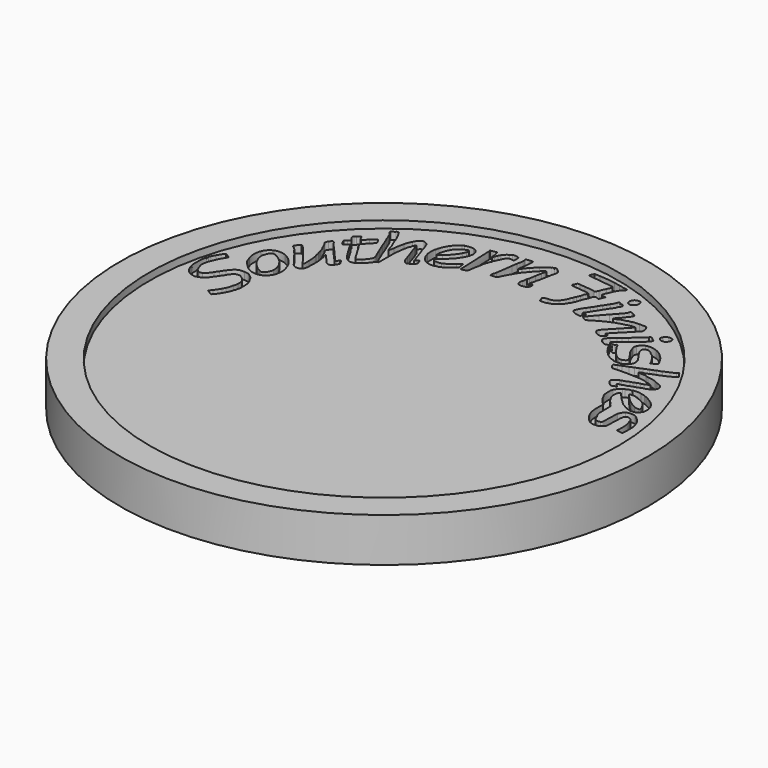
from build123d import *

# Parameters (mm, degrees)
F0_R     = 57.15
F1_DEPTH = 9.525
F2_R     = 50.8
F3_DEPTH = 1.5875
F5_DEPTH = 1.5875


# Not quite as in the source:
# - ends of sketch curves that miss each other by under 0.0002 mm in the source are joined


with BuildPart() as f1:
    # F0 (on Top) → F1 (new body)
    with BuildSketch(Plane.XY):
        Circle(F0_R)
    extrude(amount=-F1_DEPTH)

    # F2 (on Top) → F3 (cut)
    with BuildSketch(Plane.XY):
        Circle(F2_R)
    extrude(amount=-F3_DEPTH, mode=Mode.SUBTRACT)

    # F4 (on face) → F5 (cut)
    with BuildSketch(Plane.XY.offset(-1.5875)):
        with BuildLine():
            add(Edge.make_bspline(
                [(-39.9604974005, 2.8356688841), (-40.1337039629, 2.9460624826), (-40.3817034013, 3.0831555636), (-40.5116072636, 3.1403197043)],
                knots=[0, 0, 0, 0, 1, 1, 1, 1], degree=3))
            add(Edge.make_bspline(
                [(-39.5406029607, 2.6312645454), (-39.5983391878, 2.6333833838), (-39.7872908382, 2.7252752856), (-39.9604974005, 2.8356688841)],
                knots=[0, 0, 0, 0, 1, 1, 1, 1], degree=3))
            add(Edge.make_bspline(
                [(-38.7008161999, 3.6583778075), (-39.0297510269, 3.1414681147), (-39.4495183364, 2.6280650995), (-39.5406029607, 2.6312645454)],
                knots=[0, 0, 0, 0, 1, 1, 1, 1], degree=3))
            add(Edge.make_bspline(
                [(-38.3225632909, 4.2449655005), (-38.4728673291, 4.0130713527), (-38.6430799729, 3.749106467), (-38.7008161999, 3.6583778075)],
                knots=[0, 0, 0, 0, 1, 1, 1, 1], degree=3))
            add(Edge.make_bspline(
                [(-37.867599957, 5.0864833522), (-37.9675264939, 4.8555426817), (-38.1722592526, 4.4768596484), (-38.3225632909, 4.2449655005)],
                knots=[0, 0, 0, 0, 1, 1, 1, 1], degree=3))
            add(Edge.make_bspline(
                [(-37.589769393, 5.6886572204), (-37.6426534802, 5.5884022635), (-37.7676755389, 5.3174261417), (-37.867599957, 5.0864833522)],
                knots=[0, 0, 0, 0, 1, 1, 1, 1], degree=3))
            add(Edge.make_bspline(
                [(-37.4936228638, 6.0761122445), (-37.4936228638, 5.9632650312), (-37.5368895435, 5.7889100584), (-37.589769393, 5.6886572204)],
                knots=[0, 0, 0, 0, 1, 1, 1, 1], degree=3))
            add(Edge.make_bspline(
                [(-37.3886492538, 6.3461645528), (-37.446383362, 6.3104833145), (-37.4936228638, 6.1889594579), (-37.4936228638, 6.0761122445)],
                knots=[0, 0, 0, 0, 1, 1, 1, 1], degree=3))
            add(Edge.make_bspline(
                [(-37.2836756439, 6.7135711282), (-37.2836756439, 6.5471808689), (-37.3309130267, 6.38184791), (-37.3886492538, 6.3461645528)],
                knots=[0, 0, 0, 0, 1, 1, 1, 1], degree=3))
            add(Edge.make_bspline(
                [(-37.1756000545, 7.0828973712), (-37.2350419465, 7.0461588325), (-37.2836756439, 6.8799635064), (-37.2836756439, 6.7135711282)],
                knots=[0, 0, 0, 0, 1, 1, 1, 1], degree=3))
            add(Edge.make_bspline(
                [(-37.2033568373, 9.6528279692), (-37.0542753688, 9.174415451), (-37.0326377912, 7.1712508129), (-37.1756000545, 7.0828973712)],
                knots=[0, 0, 0, 0, 1, 1, 1, 1], degree=3))
            add(Edge.make_bspline(
                [(-37.6119769381, 10.5975883399), (-37.5401440793, 10.5975883399), (-37.3885221235, 10.2470265296), (-37.2033568373, 9.6528279692)],
                knots=[0, 0, 0, 0, 1, 1, 1, 1], degree=3))
            add(Edge.make_bspline(
                [(-37.7454891822, 10.7812916276), (-37.7089646462, 10.6802548194), (-37.6488849839, 10.5975883399), (-37.6119769381, 10.5975883399)],
                knots=[0, 0, 0, 0, 1, 1, 1, 1], degree=3))
            add(Edge.make_bspline(
                [(-38.9586809498, 12.2043649312), (-38.3140985315, 11.7597839054), (-37.9410049939, 11.322146313), (-37.7454891822, 10.7812916276)],
                knots=[0, 0, 0, 0, 1, 1, 1, 1], degree=3))
            add(Edge.make_bspline(
                [(-40.2763462816, 12.5716274256), (-39.5387595713, 12.5329141295), (-39.3646948794, 12.4843990871), (-38.9586809498, 12.2043649312)],
                knots=[0, 0, 0, 0, 1, 1, 1, 1], degree=3))
            add(Edge.make_bspline(
                [(-43.0340780007, 11.0498819374), (-42.0103442858, 12.3822731959), (-41.5463907207, 12.6382881999), (-40.2763462816, 12.5716274256)],
                knots=[0, 0, 0, 0, 1, 1, 1, 1], degree=3))
            add(Edge.make_bspline(
                [(-43.372132308, 10.5401190865), (-43.372132308, 10.5784997249), (-43.2200081875, 10.8078915247), (-43.0340780007, 11.0498819374)],
                knots=[0, 0, 0, 0, 1, 1, 1, 1], degree=3))
            add(Edge.make_bspline(
                [(-43.7095213001, 10.0443532819), (-43.5239576723, 10.2786459548), (-43.372132308, 10.5017405669), (-43.372132308, 10.5401190865)],
                knots=[0, 0, 0, 0, 1, 1, 1, 1], degree=3))
            add(Edge.make_bspline(
                [(-44.2442928004, 9.2500918826), (-44.1357319971, 9.4526443566), (-43.8950849279, 9.8100627278), (-43.7095213001, 10.0443532819)],
                knots=[0, 0, 0, 0, 1, 1, 1, 1], degree=3))
            add(Edge.make_bspline(
                [(-45.5492811221, 7.8108730306), (-45.1673541473, 7.9921099904), (-44.5588385959, 8.6632160276), (-44.2442928004, 9.2500918826)],
                knots=[0, 0, 0, 0, 1, 1, 1, 1], degree=3))
            add(Edge.make_bspline(
                [(-47.0540314076, 8.3486575191), (-46.4052897095, 7.6916735397), (-46.0603004442, 7.5683783343), (-45.5492811221, 7.8108730306)],
                knots=[0, 0, 0, 0, 1, 1, 1, 1], degree=3))
            Line((-47.0540314076, 8.3486575191), (-47.6132818478, 9.8690024551))
            add(Edge.make_bspline(
                [(-46.9441993012, 12.6445705557), (-47.4864503011, 11.4260753356), (-47.6015244136, 10.9487116424), (-47.6132818478, 9.8690024551)],
                knots=[0, 0, 0, 0, 1, 1, 1, 1], degree=3))
            add(Edge.make_bspline(
                [(-46.0249921214, 14.4146544964), (-46.3632307677, 13.9119855164), (-46.4816886651, 13.6838798515), (-46.9441993012, 12.6445705557)],
                knots=[0, 0, 0, 0, 1, 1, 1, 1], degree=3))
            add(Edge.make_bspline(
                [(-45.6815474893, 14.9996043273), (-45.6815474893, 14.9586026858), (-45.8360976797, 14.6953751559), (-46.0249921214, 14.4146544964)],
                knots=[0, 0, 0, 0, 1, 1, 1, 1], degree=3))
            add(Edge.make_bspline(
                [(-46.7237786632, 15.6864173134), (-46.4475457034, 15.5987440189), (-45.6815474893, 15.0939646758), (-45.6815474893, 14.9996043273)],
                knots=[0, 0, 0, 0, 1, 1, 1, 1], degree=3))
            add(Edge.make_bspline(
                [(-47.8137366717, 14.2716583317), (-47.1737436573, 15.4625472065), (-46.9467482638, 15.7571843966), (-46.7237786632, 15.6864173134)],
                knots=[0, 0, 0, 0, 1, 1, 1, 1], degree=3))
            add(Edge.make_bspline(
                [(-48.2667866945, 13.4318715709), (-48.1882583064, 13.5762089603), (-47.9843857962, 13.9541143799), (-47.8137366717, 14.2716583317)],
                knots=[0, 0, 0, 0, 1, 1, 1, 1], degree=3))
            add(Edge.make_bspline(
                [(-48.4102108646, 12.9394429368), (-48.4097870969, 13.065939707), (-48.3453150827, 13.2875320627), (-48.2667866945, 13.4318715709)],
                knots=[0, 0, 0, 0, 1, 1, 1, 1], degree=3))
            add(Edge.make_bspline(
                [(-48.5158307203, 12.6445705557), (-48.4580944932, 12.6802517941), (-48.4105668295, 12.8129461666), (-48.4102108646, 12.9394429368)],
                knots=[0, 0, 0, 0, 1, 1, 1, 1], degree=3))
            add(Edge.make_bspline(
                [(-48.6208043302, 12.2771639803), (-48.6208043302, 12.4435542396), (-48.5735669473, 12.6088871985), (-48.5158307203, 12.6445705557)],
                knots=[0, 0, 0, 0, 1, 1, 1, 1], degree=3))
            add(Edge.make_bspline(
                [(-48.7257779402, 11.9097552861), (-48.6680417131, 11.9454386432), (-48.6208043302, 12.1107716022), (-48.6208043302, 12.2771639803)],
                knots=[0, 0, 0, 0, 1, 1, 1, 1], degree=3))
            add(Edge.make_bspline(
                [(-48.7257779402, 8.865526954), (-48.8657187399, 8.9520158179), (-48.8657187399, 11.8232664221), (-48.7257779402, 11.9097552861)],
                knots=[0, 0, 0, 0, 1, 1, 1, 1], degree=3))
            add(Edge.make_bspline(
                [(-48.6208043302, 8.5600455491), (-48.6208043302, 8.6923776003), (-48.6680417131, 8.8298435968), (-48.7257779402, 8.865526954)],
                knots=[0, 0, 0, 0, 1, 1, 1, 1], degree=3))
            add(Edge.make_bspline(
                [(-47.8285960853, 6.9627338089), (-48.2123092409, 7.4696552976), (-48.6208043302, 8.2932965099), (-48.6208043302, 8.5600455491)],
                knots=[0, 0, 0, 0, 1, 1, 1, 1], degree=3))
            add(Edge.make_bspline(
                [(-46.5112019649, 6.1887051973), (-46.8499173498, 6.1887051973), (-47.5573000189, 6.6043238213), (-47.8285960853, 6.9627338089)],
                knots=[0, 0, 0, 0, 1, 1, 1, 1], degree=3))
            add(Edge.make_bspline(
                [(-46.0910829282, 6.0781865873), (-46.204659022, 6.1389718228), (-46.3937144955, 6.1887051973), (-46.5112019649, 6.1887051973)],
                knots=[0, 0, 0, 0, 1, 1, 1, 1], degree=3))
            add(Edge.make_bspline(
                [(-44.7368210199, 6.3841532062), (-45.4317872962, 6.0588585436), (-45.8699821431, 5.959857939), (-46.0910829282, 6.0781865873)],
                knots=[0, 0, 0, 0, 1, 1, 1, 1], degree=3))
            add(Edge.make_bspline(
                [(-43.1834306806, 7.9663131331), (-43.8356578678, 6.9919907293), (-44.1736125897, 6.6477769588), (-44.7368210199, 6.3841532062)],
                knots=[0, 0, 0, 0, 1, 1, 1, 1], degree=3))
            add(Edge.make_bspline(
                [(-42.4063636547, 9.0609050412), (-42.5045209616, 8.9506936627), (-42.8542013351, 8.4581273041), (-43.1834306806, 7.9663131331)],
                knots=[0, 0, 0, 0, 1, 1, 1, 1], degree=3))
            add(Edge.make_bspline(
                [(-42.0700997658, 9.5938140826), (-42.1568852671, 9.4109244288), (-42.308204229, 9.1711143008), (-42.4063636547, 9.0609050412)],
                knots=[0, 0, 0, 0, 1, 1, 1, 1], degree=3))
            add(Edge.make_bspline(
                [(-41.6974575408, 10.1207734258), (-41.8156230385, 10.0138356527), (-41.9833121457, 9.7767037363), (-42.0700997658, 9.5938140826)],
                knots=[0, 0, 0, 0, 1, 1, 1, 1], degree=3))
            add(Edge.make_bspline(
                [(-41.4826115666, 10.411410249), (-41.4826115666, 10.3584986169), (-41.5792920431, 10.2277133178), (-41.6974575408, 10.1207734258)],
                knots=[0, 0, 0, 0, 1, 1, 1, 1], degree=3))
            add(Edge.make_bspline(
                [(-40.8875633519, 10.9470038586), (-41.2546393885, 10.7571813657), (-41.4826115666, 10.5519867003), (-41.4826115666, 10.411410249)],
                knots=[0, 0, 0, 0, 1, 1, 1, 1], degree=3))
            add(Edge.make_bspline(
                [(-39.803038045, 10.8987748594), (-39.803038045, 11.0836350328), (-40.5583890963, 11.1172249777), (-40.8875633519, 10.9470038586)],
                knots=[0, 0, 0, 0, 1, 1, 1, 1], degree=3))
            add(Edge.make_bspline(
                [(-39.668017188, 10.8075355598), (-39.7422782356, 10.8075355598), (-39.803038045, 10.8485922911), (-39.803038045, 10.8987748594)],
                knots=[0, 0, 0, 0, 1, 1, 1, 1], degree=3))
            add(Edge.make_bspline(
                [(-38.5019547425, 9.6310081715), (-38.687429379, 10.0454360083), (-39.4427507666, 10.8075355598), (-39.668017188, 10.8075355598)],
                knots=[0, 0, 0, 0, 1, 1, 1, 1], degree=3))
            add(Edge.make_bspline(
                [(-38.3984388933, 8.394269753), (-38.3420502475, 9.0704228632), (-38.362980133, 9.3204818125), (-38.5019547425, 9.6310081715)],
                knots=[0, 0, 0, 0, 1, 1, 1, 1], degree=3))
            add(Edge.make_bspline(
                [(-38.5587247792, 7.4913755098), (-38.5094405985, 7.5218316927), (-38.4373132211, 7.9281359031), (-38.3984388933, 8.394269753)],
                knots=[0, 0, 0, 0, 1, 1, 1, 1], degree=3))
            add(Edge.make_bspline(
                [(-38.6483304544, 7.2095106776), (-38.6483304544, 7.334077186), (-38.6080068411, 7.4609172081), (-38.5587247792, 7.4913755098)],
                knots=[0, 0, 0, 0, 1, 1, 1, 1], degree=3))
            add(Edge.make_bspline(
                [(-39.0642499534, 5.9787579774), (-38.9541784183, 6.0761969981), (-38.6483304544, 6.9812333868), (-38.6483304544, 7.2095106776)],
                knots=[0, 0, 0, 0, 1, 1, 1, 1], degree=3))
            add(Edge.make_bspline(
                [(-39.3809781524, 5.4014041821), (-39.2393888964, 5.6900810798), (-39.0968609949, 5.9498909233), (-39.0642499534, 5.9787579774)],
                knots=[0, 0, 0, 0, 1, 1, 1, 1], degree=3))
            add(Edge.make_bspline(
                [(-40.3008167461, 4.0304225202), (-39.8815367694, 4.5217769032), (-39.6245492186, 4.9048077929), (-39.3809781524, 5.4014041821)],
                knots=[0, 0, 0, 0, 1, 1, 1, 1], degree=3))
            add(Edge.make_bspline(
                [(-40.7477984157, 3.3007623843), (-40.7477984157, 3.3924127385), (-40.4998392353, 3.7971850288), (-40.3008167461, 4.0304225202)],
                knots=[0, 0, 0, 0, 1, 1, 1, 1], degree=3))
            add(Edge.make_bspline(
                [(-40.5116072636, 3.1403197043), (-40.6415132448, 3.1974817262), (-40.7477984157, 3.2696811441), (-40.7477984157, 3.3007623843)],
                knots=[0, 0, 0, 0, 1, 1, 1, 1], degree=3))
        make_face()
        with BuildLine():
            add(Edge.make_bspline(
                [(40.1867065381, 5.8737843675), (40.1867065381, 5.9315205945), (40.0881402954, 5.9787579774), (39.9676737392, 5.9787579774)],
                knots=[0, 0, 0, 0, 1, 1, 1, 1], degree=3))
            add(Edge.make_bspline(
                [(41.82664295, 5.9222316071), (41.4789034325, 5.7487559522), (40.1867065381, 5.7105808411), (40.1867065381, 5.8737843675)],
                knots=[0, 0, 0, 0, 1, 1, 1, 1], degree=3))
            add(Edge.make_bspline(
                [(42.4463671565, 6.401211974), (42.2746649693, 6.22215318), (41.9957876992, 6.0066122268), (41.82664295, 5.9222316071)],
                knots=[0, 0, 0, 0, 1, 1, 1, 1], degree=3))
            Line((42.4463671565, 6.401211974), (42.8188737759, 8.7933953389))
            add(Edge.make_bspline(
                [(42.9563588419, 11.0733607855), (42.9139185091, 10.9560237536), (42.8520505472, 9.9300398324), (42.8188737759, 8.7933953389)],
                knots=[0, 0, 0, 0, 1, 1, 1, 1], degree=3))
            add(Edge.make_bspline(
                [(43.3277954479, 11.416957974), (43.1659458593, 11.3453158107), (42.9987991747, 11.1906978174), (42.9563588419, 11.0733607855)],
                knots=[0, 0, 0, 0, 1, 1, 1, 1], degree=3))
            add(Edge.make_bspline(
                [(44.082585007, 11.3496276468), (43.6928501128, 11.5168463719), (43.5768394737, 11.5271947785), (43.3277954479, 11.416957974)],
                knots=[0, 0, 0, 0, 1, 1, 1, 1], degree=3))
            add(Edge.make_bspline(
                [(44.7389990189, 10.5336481541), (44.559834283, 11.0992190891), (44.5037698194, 11.16891404), (44.082585007, 11.3496276468)],
                knots=[0, 0, 0, 0, 1, 1, 1, 1], degree=3))
            add(Edge.make_bspline(
                [(45.021717743, 9.7053137147), (44.9739676012, 9.82078405), (44.8467440694, 10.1935364547), (44.7389990189, 10.5336481541)],
                knots=[0, 0, 0, 0, 1, 1, 1, 1], degree=3))
            add(Edge.make_bspline(
                [(45.1758950179, 6.856173189), (45.3243810928, 7.5011327606), (45.2327159068, 9.1950931947), (45.021717743, 9.7053137147)],
                knots=[0, 0, 0, 0, 1, 1, 1, 1], degree=3))
            add(Edge.make_bspline(
                [(46.2751632022, 6.3787056727), (44.9896554806, 6.5381058842), (45.0923915972, 6.4934831478), (45.1758950179, 6.856173189)],
                knots=[0, 0, 0, 0, 1, 1, 1, 1], degree=3))
            Line((46.2751632022, 6.3787056727), (46.5671327747, 7.7052680068))
            add(Edge.make_bspline(
                [(46.5242220598, 9.2273821728), (46.5640668156, 9.1377256455), (46.5833757898, 8.4527751184), (46.5671327747, 7.7052680068)],
                knots=[0, 0, 0, 0, 1, 1, 1, 1], degree=3))
            add(Edge.make_bspline(
                [(46.4725372352, 9.4813969934), (46.4611166963, 9.4313457931), (46.4843815417, 9.3170387001), (46.5242220598, 9.2273821728)],
                knots=[0, 0, 0, 0, 1, 1, 1, 1], degree=3))
            add(Edge.make_bspline(
                [(46.0314268667, 10.8072770615), (46.2841216509, 10.2854898028), (46.5047075583, 9.6224523022), (46.4725372352, 9.4813969934)],
                knots=[0, 0, 0, 0, 1, 1, 1, 1], degree=3))
            add(Edge.make_bspline(
                [(44.2416059464, 12.6354404811), (44.7539474237, 12.4254593598), (45.7311429723, 11.4273318068), (46.0314268667, 10.8072770615)],
                knots=[0, 0, 0, 0, 1, 1, 1, 1], degree=3))
            add(Edge.make_bspline(
                [(42.2396935419, 12.581717334), (42.699333152, 12.852913815), (43.6488164135, 12.8783928465), (44.2416059464, 12.6354404811)],
                knots=[0, 0, 0, 0, 1, 1, 1, 1], degree=3))
            add(Edge.make_bspline(
                [(41.4611390915, 11.4061942751), (41.7973775543, 12.2307889646), (41.895170421, 12.378444455), (42.2396935419, 12.581717334)],
                knots=[0, 0, 0, 0, 1, 1, 1, 1], degree=3))
            add(Edge.make_bspline(
                [(41.3414141287, 9.2829020949), (41.3414141287, 10.4113742287), (41.3872975739, 11.2251013962), (41.4611390915, 11.4061942751)],
                knots=[0, 0, 0, 0, 1, 1, 1, 1], degree=3))
            add(Edge.make_bspline(
                [(41.0832463849, 7.2840683625), (41.3411429174, 7.4530478423), (41.3414141287, 7.4551454923), (41.3414141287, 9.2829020949)],
                knots=[0, 0, 0, 0, 1, 1, 1, 1], degree=3))
            add(Edge.make_bspline(
                [(39.7339362019, 7.6190990875), (39.6104672518, 7.2973450038), (40.6932063779, 7.0285046711), (41.0832463849, 7.2840683625)],
                knots=[0, 0, 0, 0, 1, 1, 1, 1], degree=3))
            add(Edge.make_bspline(
                [(39.6380799536, 7.7633051089), (39.723172503, 7.7633051089), (39.7650810073, 7.7002590729), (39.7339362019, 7.6190990875)],
                knots=[0, 0, 0, 0, 1, 1, 1, 1], degree=3))
            add(Edge.make_bspline(
                [(39.4868838843, 8.0638369073), (39.4868838843, 7.8722155206), (39.541674926, 7.7633051089), (39.6380799536, 7.7633051089)],
                knots=[0, 0, 0, 0, 1, 1, 1, 1], degree=3))
            add(Edge.make_bspline(
                [(39.2594414159, 8.6084970264), (39.3845333963, 8.4742262381), (39.4868838843, 8.2291274895), (39.4868838843, 8.0638369073)],
                knots=[0, 0, 0, 0, 1, 1, 1, 1], degree=3))
            add(Edge.make_bspline(
                [(39.0319989475, 9.0365850142), (39.0319989475, 8.9354083626), (39.1343473167, 8.7427699335), (39.2594414159, 8.6084970264)],
                knots=[0, 0, 0, 0, 1, 1, 1, 1], degree=3))
            add(Edge.make_bspline(
                [(38.9270253375, 9.2854213938), (38.9847594457, 9.2497380366), (39.0319989475, 9.1377637846), (39.0319989475, 9.0365850142)],
                knots=[0, 0, 0, 0, 1, 1, 1, 1], degree=3))
            add(Edge.make_bspline(
                [(38.8220517276, 11.1139471347), (38.8220517276, 10.0514153702), (38.8637822495, 9.3245054866), (38.9270253375, 9.2854213938)],
                knots=[0, 0, 0, 0, 1, 1, 1, 1], degree=3))
            add(Edge.make_bspline(
                [(38.5596187621, 13.0746756777), (38.8213143718, 12.8781491801), (38.8220517276, 12.8726359626), (38.8220517276, 11.1139471347)],
                knots=[0, 0, 0, 0, 1, 1, 1, 1], degree=3))
            add(Edge.make_bspline(
                [(38.2971836778, 13.3522053666), (38.2971836778, 13.3079576647), (38.4152792539, 13.1830690928), (38.5596187621, 13.0746756777)],
                knots=[0, 0, 0, 0, 1, 1, 1, 1], degree=3))
            add(Edge.make_bspline(
                [(37.8253904107, 13.9308876736), (38.0848760719, 13.6568604245), (38.2971836778, 13.3964530685), (38.2971836778, 13.3522053666)],
                knots=[0, 0, 0, 0, 1, 1, 1, 1], degree=3))
            add(Edge.make_bspline(
                [(37.3530102253, 14.5515865457), (37.3532221091, 14.4842286735), (37.5659047494, 14.2049149227), (37.8253904107, 13.9308876736)],
                knots=[0, 0, 0, 0, 1, 1, 1, 1], degree=3))
            add(Edge.make_bspline(
                [(37.260836518, 14.70904802), (37.3112097817, 14.6898089675), (37.3526881619, 14.6189444178), (37.3530102253, 14.5515865457)],
                knots=[0, 0, 0, 0, 1, 1, 1, 1], degree=3))
            add(Edge.make_bspline(
                [(36.8934278238, 15.2916586534), (37.0451281766, 14.9904678962), (37.2104611355, 14.7282913102), (37.260836518, 14.70904802)],
                knots=[0, 0, 0, 0, 1, 1, 1, 1], degree=3))
            add(Edge.make_bspline(
                [(36.7827587763, 17.299758066), (36.5237477348, 16.7805600278), (36.5704638834, 15.9328848317), (36.8934278238, 15.2916586534)],
                knots=[0, 0, 0, 0, 1, 1, 1, 1], degree=3))
            add(Edge.make_bspline(
                [(37.4164503653, 17.343192134), (37.1576999409, 17.7182816174), (36.9856629774, 17.7064902818), (36.7827587763, 17.299758066)],
                knots=[0, 0, 0, 0, 1, 1, 1, 1], degree=3))
            add(Edge.make_bspline(
                [(40.0292450637, 14.6815476167), (39.7947659331, 14.7870551739), (37.7259151863, 16.8945831964), (37.4164503653, 17.343192134)],
                knots=[0, 0, 0, 0, 1, 1, 1, 1], degree=3))
            add(Edge.make_bspline(
                [(40.9372753711, 14.1404407896), (40.4374032578, 14.4694688454), (40.2426629409, 14.5855197424), (40.0292450637, 14.6815476167)],
                knots=[0, 0, 0, 0, 1, 1, 1, 1], degree=3))
            add(Edge.make_bspline(
                [(41.383860818, 13.9567375018), (41.2917379629, 13.9567375018), (41.0907724989, 14.0394039813), (40.9372753711, 14.1404407896)],
                knots=[0, 0, 0, 0, 1, 1, 1, 1], degree=3))
            add(Edge.make_bspline(
                [(41.5513613486, 13.8517638919), (41.5513613486, 13.909500119), (41.475985792, 13.9567375018), (41.383860818, 13.9567375018)],
                knots=[0, 0, 0, 0, 1, 1, 1, 1], degree=3))
            add(Edge.make_bspline(
                [(41.8075988306, 13.7467902819), (41.6666664145, 13.7467902819), (41.5513613486, 13.7940297837), (41.5513613486, 13.8517638919)],
                knots=[0, 0, 0, 0, 1, 1, 1, 1], degree=3))
            add(Edge.make_bspline(
                [(42.1287151439, 13.641816672), (42.0930317867, 13.6995528991), (41.9485291279, 13.7467902819), (41.8075988306, 13.7467902819)],
                knots=[0, 0, 0, 0, 1, 1, 1, 1], degree=3))
            add(Edge.make_bspline(
                [(43.4685498817, 13.6680606042), (43.1885665779, 13.5115695578), (42.2209248715, 13.4926186673), (42.1287151439, 13.641816672)],
                knots=[0, 0, 0, 0, 1, 1, 1, 1], degree=3))
            add(Edge.make_bspline(
                [(44.4237603633, 14.5893124631), (44.277573228, 14.296274996), (43.8434931652, 13.8776264332), (43.4685498817, 13.6680606042)],
                knots=[0, 0, 0, 0, 1, 1, 1, 1], degree=3))
            add(Edge.make_bspline(
                [(44.4529325301, 16.2661526831), (44.5850654104, 15.8353080865), (44.568434648, 14.8793199912), (44.4237603633, 14.5893124631)],
                knots=[0, 0, 0, 0, 1, 1, 1, 1], degree=3))
            add(Edge.make_bspline(
                [(43.9132622754, 17.2824090173), (44.1382892681, 17.0370072748), (44.3234651485, 16.6883036858), (44.4529325301, 16.2661526831)],
                knots=[0, 0, 0, 0, 1, 1, 1, 1], degree=3))
            add(Edge.make_bspline(
                [(43.5153762099, 17.7801516981), (43.6187416215, 17.6323182254), (43.7977919401, 17.4083358201), (43.9132622754, 17.2824090173)],
                knots=[0, 0, 0, 0, 1, 1, 1, 1], degree=3))
            add(Edge.make_bspline(
                [(41.4463877387, 19.1424630734), (42.1142413589, 18.8745846933), (43.2926757018, 18.0986533649), (43.5153762099, 17.7801516981)],
                knots=[0, 0, 0, 0, 1, 1, 1, 1], degree=3))
            add(Edge.make_bspline(
                [(40.791728125, 19.4261310371), (40.891980963, 19.3743233199), (41.1865778951, 19.2466717827), (41.4463877387, 19.1424630734)],
                knots=[0, 0, 0, 0, 1, 1, 1, 1], degree=3))
            add(Edge.make_bspline(
                [(40.2992994909, 19.5203282351), (40.4698808125, 19.5203282351), (40.6914731681, 19.4779408732), (40.791728125, 19.4261310371)],
                knots=[0, 0, 0, 0, 1, 1, 1, 1], degree=3))
            add(Edge.make_bspline(
                [(39.9242735726, 19.625301845), (39.959954811, 19.5675677368), (40.1287160504, 19.5203282351), (40.2992994909, 19.5203282351)],
                knots=[0, 0, 0, 0, 1, 1, 1, 1], degree=3))
            add(Edge.make_bspline(
                [(38.9795110831, 19.730275455), (39.463447413, 19.730275455), (39.8885902154, 19.6830380721), (39.9242735726, 19.625301845)],
                knots=[0, 0, 0, 0, 1, 1, 1, 1], degree=3))
            add(Edge.make_bspline(
                [(38.0347507123, 19.625301845), (38.0704340695, 19.6830380721), (38.495576872, 19.730275455), (38.9795110831, 19.730275455)],
                knots=[0, 0, 0, 0, 1, 1, 1, 1], degree=3))
            add(Edge.make_bspline(
                [(37.7122105397, 19.5203282351), (37.853926926, 19.5203282351), (37.999069474, 19.5675677368), (38.0347507123, 19.625301845)],
                knots=[0, 0, 0, 0, 1, 1, 1, 1], degree=3))
            add(Edge.make_bspline(
                [(36.8275573762, 19.1888423268), (37.2888051847, 19.4492814653), (37.4784115561, 19.5203282351), (37.7122105397, 19.5203282351)],
                knots=[0, 0, 0, 0, 1, 1, 1, 1], degree=3))
            add(Edge.make_bspline(
                [(36.4601508007, 19.0050924246), (36.575621136, 19.0572561067), (36.740954095, 19.1399437746), (36.8275573762, 19.1888423268)],
                knots=[0, 0, 0, 0, 1, 1, 1, 1], degree=3))
            add(Edge.make_bspline(
                [(35.3525640569, 17.7983186184), (35.5448126198, 18.1836696361), (36.184388223, 18.8805195596), (36.4601508007, 19.0050924246)],
                knots=[0, 0, 0, 0, 1, 1, 1, 1], degree=3))
            add(Edge.make_bspline(
                [(35.5673846051, 14.9014978726), (35.2076206797, 15.1969317458), (35.0584311504, 17.2087433633), (35.3525640569, 17.7983186184)],
                knots=[0, 0, 0, 0, 1, 1, 1, 1], degree=3))
            add(Edge.make_bspline(
                [(35.8155365998, 14.4816055516), (35.7142073919, 14.6836791681), (35.6025382527, 14.8726308185), (35.5673846051, 14.9014978726)],
                knots=[0, 0, 0, 0, 1, 1, 1, 1], degree=3))
            add(Edge.make_bspline(
                [(37.0524339313, 12.8669447627), (36.473624494, 13.4259112786), (36.1009865066, 13.9123584319), (35.8155365998, 14.4816055516)],
                knots=[0, 0, 0, 0, 1, 1, 1, 1], degree=3))
            add(Edge.make_bspline(
                [(37.4600963171, 12.1247474601), (37.5705428866, 12.3311180809), (37.5290411992, 12.4066779764), (37.0524339313, 12.8669447627)],
                knots=[0, 0, 0, 0, 1, 1, 1, 1], degree=3))
            add(Edge.make_bspline(
                [(37.6779129028, 8.9180126995), (37.4608590989, 8.9180126995), (37.2674854329, 11.764850048), (37.4600963171, 12.1247474601)],
                knots=[0, 0, 0, 0, 1, 1, 1, 1], degree=3))
            add(Edge.make_bspline(
                [(37.7723177469, 8.7248339666), (37.7723177469, 8.8310831172), (37.7298350373, 8.9180126995), (37.6779129028, 8.9180126995)],
                knots=[0, 0, 0, 0, 1, 1, 1, 1], degree=3))
            add(Edge.make_bspline(
                [(38.0870033857, 7.9019089217), (37.9139260725, 8.2482690754), (37.7723177469, 8.6185848159), (37.7723177469, 8.7248339666)],
                knots=[0, 0, 0, 0, 1, 1, 1, 1], degree=3))
            add(Edge.make_bspline(
                [(39.9676737392, 5.9787579774), (39.6227395637, 5.9787579774), (38.4474474582, 7.1806012467), (38.0870033857, 7.9019089217)],
                knots=[0, 0, 0, 0, 1, 1, 1, 1], degree=3))
        make_face()
        with BuildLine():
            add(Edge.make_bspline(
                [(43.3921636392, 15.1376890247), (43.3519014722, 15.267592887), (43.2936461297, 15.4801653477), (43.2627089705, 15.61006921)],
                knots=[0, 0, 0, 0, 1, 1, 1, 1], degree=3))
            add(Edge.make_bspline(
                [(43.111962095, 14.9136748367), (43.4321609513, 14.9026356888), (43.458489637, 14.9236969423), (43.3921636392, 15.1376890247)],
                knots=[0, 0, 0, 0, 1, 1, 1, 1], degree=3))
            add(Edge.make_bspline(
                [(42.0784287526, 15.1431005379), (42.4027466307, 14.9863128542), (42.6597850336, 14.9292546554), (43.111962095, 14.9136748367)],
                knots=[0, 0, 0, 0, 1, 1, 1, 1], degree=3))
            add(Edge.make_bspline(
                [(40.6128070555, 16.0299445803), (40.6787622567, 15.9414512953), (41.6791061147, 15.336145784), (42.0784287526, 15.1431005379)],
                knots=[0, 0, 0, 0, 1, 1, 1, 1], degree=3))
            add(Edge.make_bspline(
                [(40.0292450637, 16.524869206), (40.3179219614, 16.2959710956), (40.5805244339, 16.0732557557), (40.6128070555, 16.0299445803)],
                knots=[0, 0, 0, 0, 1, 1, 1, 1], degree=3))
            add(Edge.make_bspline(
                [(39.4090314056, 17.096353819), (39.4614726556, 17.0109328497), (39.7405681661, 16.7537651976), (40.0292450637, 16.524869206)],
                knots=[0, 0, 0, 0, 1, 1, 1, 1], degree=3))
            add(Edge.make_bspline(
                [(38.9118417417, 17.6876071941), (39.1328556544, 17.447837324), (39.3565901557, 17.1817726696), (39.4090314056, 17.096353819)],
                knots=[0, 0, 0, 0, 1, 1, 1, 1], degree=3))
            add(Edge.make_bspline(
                [(38.5785484642, 18.192100494), (38.5408479729, 18.1543978838), (38.6908299477, 17.9273770643), (38.9118417417, 17.6876071941)],
                knots=[0, 0, 0, 0, 1, 1, 1, 1], degree=3))
            add(Edge.make_bspline(
                [(39.9767593182, 18.1556734245), (39.9767593182, 18.2705695546), (38.6905269538, 18.3040789836), (38.5785484642, 18.192100494)],
                knots=[0, 0, 0, 0, 1, 1, 1, 1], degree=3))
            add(Edge.make_bspline(
                [(40.291680148, 18.0507019334), (40.1184735857, 18.0507019334), (39.9767593182, 18.0979393163), (39.9767593182, 18.1556734245)],
                knots=[0, 0, 0, 0, 1, 1, 1, 1], degree=3))
            add(Edge.make_bspline(
                [(40.6065988591, 17.9457283235), (40.6065988591, 18.0034624317), (40.4648845916, 18.0507019334), (40.291680148, 18.0507019334)],
                knots=[0, 0, 0, 0, 1, 1, 1, 1], degree=3))
            add(Edge.make_bspline(
                [(40.7683594565, 17.8407547135), (40.6793915517, 17.8407547135), (40.6065988591, 17.8879920964), (40.6065988591, 17.9457283235)],
                knots=[0, 0, 0, 0, 1, 1, 1, 1], degree=3))
            add(Edge.make_bspline(
                [(41.5507447666, 17.5177526341), (41.2094020222, 17.6954045194), (40.8573273613, 17.8407547135), (40.7683594565, 17.8407547135)],
                knots=[0, 0, 0, 0, 1, 1, 1, 1], degree=3))
            add(Edge.make_bspline(
                [(42.977216687, 16.1113397567), (42.8721943437, 16.5297827922), (42.227224178, 17.1656843297), (41.5507447666, 17.5177526341)],
                knots=[0, 0, 0, 0, 1, 1, 1, 1], degree=3))
            add(Edge.make_bspline(
                [(43.1251031307, 15.8462582433), (43.0803575017, 15.8462582433), (43.0138090258, 15.9655467254), (42.977216687, 16.1113397567)],
                knots=[0, 0, 0, 0, 1, 1, 1, 1], degree=3))
            add(Edge.make_bspline(
                [(43.2627089705, 15.61006921), (43.2317718113, 15.7399730724), (43.1698508785, 15.8462582433), (43.1251031307, 15.8462582433)],
                knots=[0, 0, 0, 0, 1, 1, 1, 1], degree=3))
        make_face(mode=Mode.SUBTRACT)
        Polygon((42.8188737759, 8.7933953389), (42.4463671565, 6.401211974), (42.7585546848, 6.7267693725), align=None)
        Polygon((46.5671327747, 7.7052680068), (46.2751632022, 6.3787056727), (46.5375982865, 6.3461645528), align=None)
        with BuildLine():
            add(Edge.make_bspline(
                [(-38.7533040643, 13.1990642037), (-39.4793197982, 13.2446001594), (-40.3914013246, 13.7472988032), (-41.2201786011, 14.5586952484)],
                knots=[0, 0, 0, 0, 1, 1, 1, 1], degree=3))
            add(Edge.make_bspline(
                [(-37.8694772478, 13.2084040433), (-38.0957713058, 13.1869719931), (-38.4934942208, 13.1827703366), (-38.7533040643, 13.1990642037)],
                knots=[0, 0, 0, 0, 1, 1, 1, 1], degree=3))
            add(Edge.make_bspline(
                [(-36.2864274087, 14.0269769942), (-36.4376467852, 13.7453748979), (-37.387899185, 13.2540120395), (-37.8694772478, 13.2084040433)],
                knots=[0, 0, 0, 0, 1, 1, 1, 1], degree=3))
            add(Edge.make_bspline(
                [(-35.9061933858, 14.5882233801), (-36.057586507, 14.3870545077), (-36.2286933005, 14.1344953291), (-36.2864274087, 14.0269769942)],
                knots=[0, 0, 0, 0, 1, 1, 1, 1], degree=3))
            add(Edge.make_bspline(
                [(-35.4248399199, 16.3681938207), (-35.488710184, 15.3438138601), (-35.5734870265, 15.0303147708), (-35.9061933858, 14.5882233801)],
                knots=[0, 0, 0, 0, 1, 1, 1, 1], degree=3))
            add(Edge.make_bspline(
                [(-35.719305484, 18.1804934974), (-35.4804869723, 17.7210191566), (-35.3793166772, 17.098360359), (-35.4248399199, 16.3681938207)],
                knots=[0, 0, 0, 0, 1, 1, 1, 1], degree=3))
            add(Edge.make_bspline(
                [(-35.8140472234, 18.5084345891), (-35.8140472234, 18.4283213098), (-35.7714140763, 18.2807463354), (-35.719305484, 18.1804934974)],
                knots=[0, 0, 0, 0, 1, 1, 1, 1], degree=3))
            add(Edge.make_bspline(
                [(-36.0739969102, 19.113456176), (-35.9310240528, 18.860810125), (-35.8140472234, 18.5885499871), (-35.8140472234, 18.5084345891)],
                knots=[0, 0, 0, 0, 1, 1, 1, 1], degree=3))
            add(Edge.make_bspline(
                [(-38.7533040643, 21.6918091565), (-37.6308918083, 21.1609786955), (-36.7565298428, 20.3195604292), (-36.0739969102, 19.113456176)],
                knots=[0, 0, 0, 0, 1, 1, 1, 1], degree=3))
            add(Edge.make_bspline(
                [(-41.2987069892, 21.797365447), (-40.6864114301, 22.0887332694), (-39.4874434246, 22.039012608), (-38.7533040643, 21.6918091565)],
                knots=[0, 0, 0, 0, 1, 1, 1, 1], degree=3))
            add(Edge.make_bspline(
                [(-42.6373191572, 20.6333053038), (-42.6373191572, 20.7893619883), (-41.6950505404, 21.6087591673), (-41.2987069892, 21.797365447)],
                knots=[0, 0, 0, 0, 1, 1, 1, 1], degree=3))
            add(Edge.make_bspline(
                [(-42.7847627637, 20.2185215021), (-42.7036684623, 20.4004513221), (-42.6373191572, 20.5871061517), (-42.6373191572, 20.6333053038)],
                knots=[0, 0, 0, 0, 1, 1, 1, 1], degree=3))
            add(Edge.make_bspline(
                [(-42.8489105957, 17.1584273083), (-43.1764999602, 17.919973843), (-43.1452704013, 19.4097397034), (-42.7847627637, 20.2185215021)],
                knots=[0, 0, 0, 0, 1, 1, 1, 1], degree=3))
            add(Edge.make_bspline(
                [(-42.5721161437, 16.4236120386), (-42.6746806344, 16.7122889363), (-42.7992386675, 17.042956973), (-42.8489105957, 17.1584273083)],
                knots=[0, 0, 0, 0, 1, 1, 1, 1], degree=3))
            add(Edge.make_bspline(
                [(-41.2201786011, 14.5586952484), (-42.1005665429, 15.4206196326), (-42.3264834477, 15.7322583818), (-42.5721161437, 16.4236120386)],
                knots=[0, 0, 0, 0, 1, 1, 1, 1], degree=3))
        make_face()
        with BuildLine():
            add(Edge.make_bspline(
                [(-37.7775641576, 14.393211852), (-37.652645922, 14.4600633218), (-37.4997780893, 14.5663506115), (-37.4378571564, 14.6294008853)],
                knots=[0, 0, 0, 0, 1, 1, 1, 1], degree=3))
            add(Edge.make_bspline(
                [(-38.59584259, 14.5371530186), (-38.0965234934, 14.2415644702), (-38.0697265444, 14.2368500548), (-37.7775641576, 14.393211852)],
                knots=[0, 0, 0, 0, 1, 1, 1, 1], degree=3))
            add(Edge.make_bspline(
                [(-39.2256842497, 14.8869668789), (-39.1102117956, 14.8312816874), (-38.8267853794, 14.6738668275), (-38.59584259, 14.5371530186)],
                knots=[0, 0, 0, 0, 1, 1, 1, 1], degree=3))
            add(Edge.make_bspline(
                [(-40.9562688053, 16.6902699678), (-40.7177236237, 16.2690893931), (-39.5340303241, 15.0356606001), (-39.2256842497, 14.8869668789)],
                knots=[0, 0, 0, 0, 1, 1, 1, 1], degree=3))
            add(Edge.make_bspline(
                [(-41.6925587865, 18.9179890976), (-41.6925587865, 18.2669823613), (-41.4729475447, 17.6025273577), (-40.9562688053, 16.6902699678)],
                knots=[0, 0, 0, 0, 1, 1, 1, 1], degree=3))
            add(Edge.make_bspline(
                [(-41.5875851765, 19.4678424895), (-41.6453214036, 19.4321591323), (-41.6925587865, 19.1847254238), (-41.6925587865, 18.9179890976)],
                knots=[0, 0, 0, 0, 1, 1, 1, 1], degree=3))
            add(Edge.make_bspline(
                [(-41.4826115666, 19.7291927286), (-41.4826115666, 19.6211319711), (-41.5298489494, 19.5035237279), (-41.5875851765, 19.4678424895)],
                knots=[0, 0, 0, 0, 1, 1, 1, 1], degree=3))
            add(Edge.make_bspline(
                [(-40.791490982, 20.7611199915), (-41.0570344022, 20.6355194899), (-41.4826115666, 20.000081978), (-41.4826115666, 19.7291927286)],
                knots=[0, 0, 0, 0, 1, 1, 1, 1], degree=3))
            add(Edge.make_bspline(
                [(-39.803038045, 20.5443776569), (-39.803038045, 20.7018582008), (-40.5640018991, 20.8687188422), (-40.791490982, 20.7611199915)],
                knots=[0, 0, 0, 0, 1, 1, 1, 1], degree=3))
            add(Edge.make_bspline(
                [(-39.6907353731, 20.4650886058), (-39.7525016308, 20.4650886058), (-39.803038045, 20.5007698442), (-39.803038045, 20.5443776569)],
                knots=[0, 0, 0, 0, 1, 1, 1, 1], degree=3))
            add(Edge.make_bspline(
                [(-38.3771699936, 19.5584376622), (-38.7949561892, 19.9463990888), (-39.5464382416, 20.4650886058), (-39.6907353731, 20.4650886058)],
                knots=[0, 0, 0, 0, 1, 1, 1, 1], degree=3))
            add(Edge.make_bspline(
                [(-37.5461086093, 18.4825635724), (-37.8858791757, 19.028043682), (-38.08855878, 19.290430033), (-38.3771699936, 19.5584376622)],
                knots=[0, 0, 0, 0, 1, 1, 1, 1], degree=3))
            add(Edge.make_bspline(
                [(-37.2695048528, 18.0511511272), (-37.3639012215, 18.1957364207), (-37.4883723822, 18.3898728686), (-37.5461086093, 18.4825635724)],
                knots=[0, 0, 0, 0, 1, 1, 1, 1], degree=3))
            add(Edge.make_bspline(
                [(-36.8283118495, 16.1155287002), (-36.7745039488, 16.6038171241), (-37.0158396405, 17.6626091389), (-37.2695048528, 18.0511511272)],
                knots=[0, 0, 0, 0, 1, 1, 1, 1], degree=3))
            add(Edge.make_bspline(
                [(-37.4378571564, 14.6294008853), (-37.22035204, 14.8508767048), (-36.8748436592, 15.6932526861), (-36.8283118495, 16.1155287002)],
                knots=[0, 0, 0, 0, 1, 1, 1, 1], degree=3))
        make_face(mode=Mode.SUBTRACT)
        with BuildLine():
            add(Edge.make_bspline(
                [(33.5845332706, 19.0627947503), (33.1402954966, 19.4521969869), (32.8385665545, 19.9405892339), (32.8385665545, 20.2702508224)],
                knots=[0, 0, 0, 0, 1, 1, 1, 1], degree=3))
            add(Edge.make_bspline(
                [(34.3431325011, 18.7540312647), (34.0634564289, 18.6995516923), (33.942998348, 18.7485858501), (33.5845332706, 19.0627947503)],
                knots=[0, 0, 0, 0, 1, 1, 1, 1], degree=3))
            add(Edge.make_bspline(
                [(34.7105920475, 18.907127932), (34.6913529949, 18.8585450868), (34.5259903723, 18.7896510568), (34.3431325011, 18.7540312647)],
                knots=[0, 0, 0, 0, 1, 1, 1, 1], degree=3))
            add(Edge.make_bspline(
                [(35.0255128773, 18.9998313489), (34.871551724, 18.9974370615), (34.7298374565, 18.9557107773), (34.7105920475, 18.907127932)],
                knots=[0, 0, 0, 0, 1, 1, 1, 1], degree=3))
            add(Edge.make_bspline(
                [(34.901664655, 19.3608750527), (35.3051847118, 19.0044271094), (35.3052631089, 19.0041982748), (35.0255128773, 18.9998313489)],
                knots=[0, 0, 0, 0, 1, 1, 1, 1], degree=3))
            add(Edge.make_bspline(
                [(34.5629471513, 19.822819959), (34.5271620899, 19.7649205814), (34.6795849666, 19.5570455854), (34.901664655, 19.3608750527)],
                knots=[0, 0, 0, 0, 1, 1, 1, 1], degree=3))
            add(Edge.make_bspline(
                [(35.0992336211, 19.9987555852), (34.8400594291, 19.9598918516), (34.5987300939, 19.8807193366), (34.5629471513, 19.822819959)],
                knots=[0, 0, 0, 0, 1, 1, 1, 1], degree=3))
            add(Edge.make_bspline(
                [(35.6278477771, 20.162281175), (35.5962834418, 20.1112086946), (35.3584056943, 20.0376214376), (35.0992336211, 19.9987555852)],
                knots=[0, 0, 0, 0, 1, 1, 1, 1], degree=3))
            add(Edge.make_bspline(
                [(35.8904163483, 20.2551435047), (35.7775691349, 20.2551435047), (35.6594142314, 20.2133557742), (35.6278477771, 20.162281175)],
                knots=[0, 0, 0, 0, 1, 1, 1, 1], degree=3))
            add(Edge.make_bspline(
                [(36.2778713724, 20.34786811), (36.1776164156, 20.296869789), (36.0032614428, 20.2551435047), (35.8904163483, 20.2551435047)],
                knots=[0, 0, 0, 0, 1, 1, 1, 1], degree=3))
            add(Edge.make_bspline(
                [(37.562370527, 20.8378452481), (37.0019144678, 20.6719359652), (36.6541219793, 20.5392691375), (36.2778713724, 20.34786811)],
                knots=[0, 0, 0, 0, 1, 1, 1, 1], degree=3))
            add(Edge.make_bspline(
                [(38.8468696815, 21.3171243713), (38.5147608347, 21.1481787929), (38.1463774748, 21.0107255094), (37.562370527, 20.8378452481)],
                knots=[0, 0, 0, 0, 1, 1, 1, 1], degree=3))
            add(Edge.make_bspline(
                [(39.2343247057, 21.4098510954), (39.1214796112, 21.4098510954), (38.9471246384, 21.3681226923), (38.8468696815, 21.3171243713)],
                knots=[0, 0, 0, 0, 1, 1, 1, 1], degree=3))
            add(Edge.make_bspline(
                [(39.4987324285, 21.5056903931), (39.4661552884, 21.4529779318), (39.3471719191, 21.4098510954), (39.2343247057, 21.4098510954)],
                knots=[0, 0, 0, 0, 1, 1, 1, 1], degree=3))
            add(Edge.make_bspline(
                [(39.9707396983, 21.6712670184), (39.7437146411, 21.632911806), (39.5313116875, 21.5584007355), (39.4987324285, 21.5056903931)],
                knots=[0, 0, 0, 0, 1, 1, 1, 1], degree=3))
            add(Edge.make_bspline(
                [(40.9215196889, 22.4335763349), (40.9215196889, 22.1401214567), (40.4344623101, 21.7496131864), (39.9707396983, 21.6712670184)],
                knots=[0, 0, 0, 0, 1, 1, 1, 1], degree=3))
            add(Edge.make_bspline(
                [(41.0398017227, 22.7458231907), (40.9747470279, 22.6807684959), (40.9215196889, 22.5402577286), (40.9215196889, 22.4335763349)],
                knots=[0, 0, 0, 0, 1, 1, 1, 1], degree=3))
            add(Edge.make_bspline(
                [(41.0923192509, 23.1261356107), (41.1286276654, 22.9814698014), (41.1050958463, 22.8111279085), (41.0398017227, 22.7458231907)],
                knots=[0, 0, 0, 0, 1, 1, 1, 1], degree=3))
            add(Edge.make_bspline(
                [(40.3715412855, 24.0341849876), (40.5358275383, 24.0341849876), (41.0163525384, 23.4288095547), (41.0923192509, 23.1261356107)],
                knots=[0, 0, 0, 0, 1, 1, 1, 1], degree=3))
            add(Edge.make_bspline(
                [(39.6723013123, 24.3076210808), (39.9956000291, 24.157232289), (40.310258123, 24.0341849876), (40.3715412855, 24.0341849876)],
                knots=[0, 0, 0, 0, 1, 1, 1, 1], degree=3))
            add(Edge.make_bspline(
                [(38.8745374731, 24.6689063321), (38.9900099272, 24.6205883417), (39.3490025954, 24.4580098726), (39.6723013123, 24.3076210808)],
                knots=[0, 0, 0, 0, 1, 1, 1, 1], degree=3))
            add(Edge.make_bspline(
                [(37.1424760872, 25.0521639375), (37.6866403981, 24.9921351273), (38.5683038806, 24.797047321), (38.8745374731, 24.6689063321)],
                knots=[0, 0, 0, 0, 1, 1, 1, 1], degree=3))
            add(Edge.make_bspline(
                [(36.5703727734, 25.199069359), (36.6252210237, 25.1469332218), (36.8826683625, 25.0808254643), (37.1424760872, 25.0521639375)],
                knots=[0, 0, 0, 0, 1, 1, 1, 1], degree=3))
            add(Edge.make_bspline(
                [(35.651854216, 25.2938661882), (36.1021900068, 25.2938661882), (36.5155224042, 25.2512076151), (36.5703727734, 25.199069359)],
                knots=[0, 0, 0, 0, 1, 1, 1, 1], degree=3))
            add(Edge.make_bspline(
                [(34.8330609059, 25.3868789555), (34.8330609059, 25.3357217216), (35.2015184252, 25.2938661882), (35.651854216, 25.2938661882)],
                knots=[0, 0, 0, 0, 1, 1, 1, 1], degree=3))
            add(Edge.make_bspline(
                [(35.6988288629, 25.818734238), (35.4792917805, 25.818734238), (34.8330609059, 25.4963868796), (34.8330609059, 25.3868789555)],
                knots=[0, 0, 0, 0, 1, 1, 1, 1], degree=3))
            add(Edge.make_bspline(
                [(36.1553453053, 25.9647455097), (35.9877028126, 25.8844394162), (35.7822708372, 25.818734238), (35.6988288629, 25.818734238)],
                knots=[0, 0, 0, 0, 1, 1, 1, 1], degree=3))
            add(Edge.make_bspline(
                [(37.457396917, 26.4995509115), (37.1966653788, 26.4323201696), (36.7390280709, 26.2443495414), (36.1553453053, 25.9647455097)],
                knots=[0, 0, 0, 0, 1, 1, 1, 1], degree=3))
            add(Edge.make_bspline(
                [(38.1922121867, 26.783627811), (37.9324023431, 26.6646041837), (37.6017364253, 26.5367683076), (37.457396917, 26.4995509115)],
                knots=[0, 0, 0, 0, 1, 1, 1, 1], degree=3))
            add(Edge.make_bspline(
                [(38.8745374731, 27.0753749055), (38.7590671378, 27.0339389021), (38.4520199114, 26.9026535571), (38.1922121867, 26.783627811)],
                knots=[0, 0, 0, 0, 1, 1, 1, 1], degree=3))
            add(Edge.make_bspline(
                [(40.3949269047, 27.8394725216), (40.3934437178, 27.7673048863), (39.3711020798, 27.253560738), (38.8745374731, 27.0753749055)],
                knots=[0, 0, 0, 0, 1, 1, 1, 1], degree=3))
            add(Edge.make_bspline(
                [(40.5278691813, 27.9205371592), (40.4556994272, 27.9192658562), (40.3958761443, 27.8827731027), (40.3949269047, 27.8394725216)],
                knots=[0, 0, 0, 0, 1, 1, 1, 1], degree=3))
            add(Edge.make_bspline(
                [(40.9111564504, 28.1166695529), (40.7725166174, 28.0100792692), (40.6000389354, 27.9218211753), (40.5278691813, 27.9205371592)],
                knots=[0, 0, 0, 0, 1, 1, 1, 1], degree=3))
            Line((40.9111564504, 28.1166695529), (40.858668586, 28.7179323205))
            add(Edge.make_bspline(
                [(40.4753834357, 29.1603881514), (40.5186840169, 29.1411490989), (40.6911638177, 28.9420376185), (40.858668586, 28.7179323205)],
                knots=[0, 0, 0, 0, 1, 1, 1, 1], degree=3))
            add(Edge.make_bspline(
                [(40.396653758, 29.3378959557), (40.396653758, 29.2595116486), (40.4320807357, 29.1796335604), (40.4753834357, 29.1603881514)],
                knots=[0, 0, 0, 0, 1, 1, 1, 1], degree=3))
            add(Edge.make_bspline(
                [(39.8364710289, 29.3064100173), (40.1597845776, 29.6130483079), (40.396653758, 29.6263630883), (40.396653758, 29.3378959557)],
                knots=[0, 0, 0, 0, 1, 1, 1, 1], degree=3))
            add(Edge.make_bspline(
                [(38.6698047145, 28.6530153501), (38.9231351502, 28.6530153501), (39.47116846, 28.9599418028), (39.8364710289, 29.3064100173)],
                knots=[0, 0, 0, 0, 1, 1, 1, 1], degree=3))
            add(Edge.make_bspline(
                [(38.5071308977, 28.5480417402), (38.5071308977, 28.6057779673), (38.580334645, 28.6530153501), (38.6698047145, 28.6530153501)],
                knots=[0, 0, 0, 0, 1, 1, 1, 1], degree=3))
            add(Edge.make_bspline(
                [(38.3003788861, 28.4430681302), (38.4140927044, 28.4430681302), (38.5071308977, 28.490307632), (38.5071308977, 28.5480417402)],
                knots=[0, 0, 0, 0, 1, 1, 1, 1], degree=3))
            add(Edge.make_bspline(
                [(37.7198298825, 28.2331230292), (37.925416533, 28.3485933645), (38.186662949, 28.4430681302), (38.3003788861, 28.4430681302)],
                knots=[0, 0, 0, 0, 1, 1, 1, 1], degree=3))
            add(Edge.make_bspline(
                [(37.2338785373, 28.0231758093), (37.2955663979, 28.0231758093), (37.5142453508, 28.117650575), (37.7198298825, 28.2331230292)],
                knots=[0, 0, 0, 0, 1, 1, 1, 1], degree=3))
            add(Edge.make_bspline(
                [(36.7384475092, 27.8550120823), (36.9492465021, 27.9475014965), (37.1721906766, 28.0231758093), (37.2338785373, 28.0231758093)],
                knots=[0, 0, 0, 0, 1, 1, 1, 1], degree=3))
            add(Edge.make_bspline(
                [(36.1452299709, 27.6032813695), (36.2607003062, 27.6492432116), (36.5276485162, 27.7625226681), (36.7384475092, 27.8550120823)],
                knots=[0, 0, 0, 0, 1, 1, 1, 1], degree=3))
            add(Edge.make_bspline(
                [(35.5520103138, 27.3515506567), (35.7628093067, 27.4440421897), (36.0297596356, 27.5573195273), (36.1452299709, 27.6032813695)],
                knots=[0, 0, 0, 0, 1, 1, 1, 1], degree=3))
            add(Edge.make_bspline(
                [(35.1047298879, 27.1833890485), (35.1399365064, 27.1833890485), (35.3412113208, 27.2590612425), (35.5520103138, 27.3515506567)],
                knots=[0, 0, 0, 0, 1, 1, 1, 1], degree=3))
            add(Edge.make_bspline(
                [(34.5432398355, 26.9629790047), (34.81685603, 27.084204105), (35.0695253882, 27.1833890485), (35.1047298879, 27.1833890485)],
                knots=[0, 0, 0, 0, 1, 1, 1, 1], degree=3))
            add(Edge.make_bspline(
                [(33.8358147896, 26.6606250053), (33.9512851249, 26.7056969353), (34.2696278788, 26.8417560232), (34.5432398355, 26.9629790047)],
                knots=[0, 0, 0, 0, 1, 1, 1, 1], degree=3))
            add(Edge.make_bspline(
                [(33.1534873844, 26.3942806641), (33.4132972279, 26.4957009821), (33.7203444543, 26.6155573129), (33.8358147896, 26.6606250053)],
                knots=[0, 0, 0, 0, 1, 1, 1, 1], degree=3))
            add(Edge.make_bspline(
                [(32.2361129997, 26.0143072583), (32.4808600212, 26.1218722076), (32.8936775408, 26.2928603462), (33.1534873844, 26.3942806641)],
                knots=[0, 0, 0, 0, 1, 1, 1, 1], degree=3))
            add(Edge.make_bspline(
                [(31.6325173911, 25.818734238), (31.7197478484, 25.818734238), (31.9913680971, 25.906742309), (32.2361129997, 26.0143072583)],
                knots=[0, 0, 0, 0, 1, 1, 1, 1], degree=3))
            add(Edge.make_bspline(
                [(31.473911744, 25.7185174202), (31.473911744, 25.7736368818), (31.5452848149, 25.818734238), (31.6325173911, 25.818734238)],
                knots=[0, 0, 0, 0, 1, 1, 1, 1], degree=3))
            add(Edge.make_bspline(
                [(31.0802612364, 25.544482392), (31.2967704988, 25.5850835731), (31.473911744, 25.6633979585), (31.473911744, 25.7185174202)],
                knots=[0, 0, 0, 0, 1, 1, 1, 1], degree=3))
            add(Edge.make_bspline(
                [(30.3422549961, 25.2772926344), (30.5316516026, 25.383647727), (30.8637540929, 25.5038833298), (31.0802612364, 25.544482392)],
                knots=[0, 0, 0, 0, 1, 1, 1, 1], degree=3))
            add(Edge.make_bspline(
                [(29.8403382037, 25.0839189683), (29.9269965747, 25.0839189683), (30.1528583897, 25.1709375418), (30.3422549961, 25.2772926344)],
                knots=[0, 0, 0, 0, 1, 1, 1, 1], degree=3))
            add(Edge.make_bspline(
                [(29.9185932617, 24.3080554427), (29.5713876914, 24.7899746384), (29.5417387859, 25.0839189683), (29.8403382037, 25.0839189683)],
                knots=[0, 0, 0, 0, 1, 1, 1, 1], degree=3))
            add(Edge.make_bspline(
                [(30.6866128476, 23.8906718264), (30.2810205669, 23.8271045561), (30.2548613882, 23.8413198428), (29.9185932617, 24.3080554427)],
                knots=[0, 0, 0, 0, 1, 1, 1, 1], degree=3))
            add(Edge.make_bspline(
                [(36.1977157165, 23.8400654904), (35.4704583433, 23.9633373887), (31.3893700926, 24.0008132831), (30.6866128476, 23.8906718264)],
                knots=[0, 0, 0, 0, 1, 1, 1, 1], degree=3))
            add(Edge.make_bspline(
                [(37.3261814937, 23.6583242471), (37.0808051772, 23.6946708007), (36.5729958953, 23.7764537245), (36.1977157165, 23.8400654904)],
                knots=[0, 0, 0, 0, 1, 1, 1, 1], degree=3))
            add(Edge.make_bspline(
                [(37.7723177469, 23.5125608794), (37.7723177469, 23.5563848137), (37.5715556914, 23.6219776935), (37.3261814937, 23.6583242471)],
                knots=[0, 0, 0, 0, 1, 1, 1, 1], degree=3))
            add(Edge.make_bspline(
                [(38.2313301809, 23.369967294), (37.9788727065, 23.4045700436), (37.7723177469, 23.4687369452), (37.7723177469, 23.5125608794)],
                knots=[0, 0, 0, 0, 1, 1, 1, 1], degree=3))
            add(Edge.make_bspline(
                [(39.0305729692, 22.879477397), (39.6163025327, 22.879477397), (38.9854968015, 23.2665976447), (38.2313301809, 23.369967294)],
                knots=[0, 0, 0, 0, 1, 1, 1, 1], degree=3))
            add(Edge.make_bspline(
                [(38.2406615451, 22.593925786), (38.7414511155, 22.847580404), (38.8296922588, 22.879477397), (39.0305729692, 22.879477397)],
                knots=[0, 0, 0, 0, 1, 1, 1, 1], degree=3))
            add(Edge.make_bspline(
                [(37.562370527, 22.4070972116), (37.8177392853, 22.4502409988), (38.1229706672, 22.5343143869), (38.2406615451, 22.593925786)],
                knots=[0, 0, 0, 0, 1, 1, 1, 1], degree=3))
            add(Edge.make_bspline(
                [(36.910323441, 22.2366578522), (37.0135807919, 22.2872557128), (37.3070017687, 22.3639534245), (37.562370527, 22.4070972116)],
                knots=[0, 0, 0, 0, 1, 1, 1, 1], degree=3))
            add(Edge.make_bspline(
                [(36.5140604057, 22.0396906362), (36.6287488896, 22.0974268633), (36.8070660902, 22.1860621105), (36.910323441, 22.2366578522)],
                knots=[0, 0, 0, 0, 1, 1, 1, 1], degree=3))
            add(Edge.make_bspline(
                [(36.1452299709, 21.9347170263), (36.2333990736, 21.9347170263), (36.3993740406, 21.9819544092), (36.5140604057, 22.0396906362)],
                knots=[0, 0, 0, 0, 1, 1, 1, 1], degree=3))
            add(Edge.make_bspline(
                [(35.8026413495, 21.8385683782), (35.9028941875, 21.8914503465), (36.0570587493, 21.9347170263), (36.1452299709, 21.9347170263)],
                knots=[0, 0, 0, 0, 1, 1, 1, 1], degree=3))
            add(Edge.make_bspline(
                [(34.6396893587, 21.4098510954), (34.8356967409, 21.4098510954), (35.3477140358, 21.5986035749), (35.8026413495, 21.8385683782)],
                knots=[0, 0, 0, 0, 1, 1, 1, 1], degree=3))
            add(Edge.make_bspline(
                [(34.3606807206, 21.3048774854), (34.3963640777, 21.3626115936), (34.5219179649, 21.4098510954), (34.6396893587, 21.4098510954)],
                knots=[0, 0, 0, 0, 1, 1, 1, 1], degree=3))
            add(Edge.make_bspline(
                [(34.0658083395, 21.1973019419), (34.1923072285, 21.1987851288), (34.3249994822, 21.2471412583), (34.3606807206, 21.3048774854)],
                knots=[0, 0, 0, 0, 1, 1, 1, 1], degree=3))
            add(Edge.make_bspline(
                [(32.8385665545, 20.2702508224), (32.8385665545, 20.5072174693), (33.7473405742, 21.1936977978), (34.0658083395, 21.1973019419)],
                knots=[0, 0, 0, 0, 1, 1, 1, 1], degree=3))
        make_face()
        Polygon((40.858668586, 28.7179323205), (40.9111564504, 28.1166695529), (41.1632240585, 28.3104669866), align=None)
        with BuildLine():
            add(Edge.make_bspline(
                [(-34.6593396327, 19.283022574), (-34.9257538955, 19.3284843703), (-35.6041000035, 19.9002274816), (-35.6041000035, 20.0793095828)],
                knots=[0, 0, 0, 0, 1, 1, 1, 1], degree=3))
            add(Edge.make_bspline(
                [(-33.4812082838, 19.4890393487), (-33.6938337154, 19.296617041), (-34.2100335974, 19.2063481695), (-34.6593396327, 19.283022574)],
                knots=[0, 0, 0, 0, 1, 1, 1, 1], degree=3))
            add(Edge.make_bspline(
                [(-32.9469474235, 22.1446642462), (-32.9563550659, 20.3228340345), (-33.0446089222, 19.8841582113), (-33.4812082838, 19.4890393487)],
                knots=[0, 0, 0, 0, 1, 1, 1, 1], degree=3))
            add(Edge.make_bspline(
                [(-33.4269278821, 25.6873577829), (-33.0920115745, 24.9878677868), (-32.9381330558, 23.8520983736), (-32.9469474235, 22.1446642462)],
                knots=[0, 0, 0, 0, 1, 1, 1, 1], degree=3))
            add(Edge.make_bspline(
                [(-33.3110697994, 25.9502187538), (-33.4441731077, 26.1655838434), (-33.5456569909, 25.9353445083), (-33.4269278821, 25.6873577829)],
                knots=[0, 0, 0, 0, 1, 1, 1, 1], degree=3))
            add(Edge.make_bspline(
                [(-31.7200849106, 24.0315661034), (-32.1742430859, 24.5361865336), (-33.2065453832, 25.7810930741), (-33.3110697994, 25.9502187538)],
                knots=[0, 0, 0, 0, 1, 1, 1, 1], degree=3))
            add(Edge.make_bspline(
                [(-30.2683945759, 23.7727669458), (-30.7286931448, 23.3854517649), (-31.2169137659, 23.472489408), (-31.7200849106, 24.0315661034)],
                knots=[0, 0, 0, 0, 1, 1, 1, 1], degree=3))
            add(Edge.make_bspline(
                [(-29.9355356603, 24.2009778262), (-29.9355356603, 24.1195063716), (-30.085322702, 23.9268107338), (-30.2683945759, 23.7727669458)],
                knots=[0, 0, 0, 0, 1, 1, 1, 1], degree=3))
            add(Edge.make_bspline(
                [(-29.8568059825, 24.3499236891), (-29.9001065637, 24.3494999214), (-29.9355356603, 24.282447162), (-29.9355356603, 24.2009778262)],
                knots=[0, 0, 0, 0, 1, 1, 1, 1], degree=3))
            add(Edge.make_bspline(
                [(-29.5156433393, 25.0316811268), (-29.5156433393, 24.8547369336), (-29.7677978198, 24.3508496215), (-29.8568059825, 24.3499236891)],
                knots=[0, 0, 0, 0, 1, 1, 1, 1], degree=3))
            add(Edge.make_bspline(
                [(-29.8420715804, 25.5914083057), (-29.6625360478, 25.3472778661), (-29.5156433393, 25.0953988347), (-29.5156433393, 25.0316811268)],
                knots=[0, 0, 0, 0, 1, 1, 1, 1], degree=3))
            add(Edge.make_bspline(
                [(-30.3144517658, 25.9141561245), (-30.1976995333, 26.0110506037), (-30.1031993414, 25.9464853605), (-29.8420715804, 25.5914083057)],
                knots=[0, 0, 0, 0, 1, 1, 1, 1], degree=3))
            add(Edge.make_bspline(
                [(-30.46040371, 25.6612727636), (-30.46040371, 25.7337370363), (-30.3947260767, 25.8475334893), (-30.3144517658, 25.9141561245)],
                knots=[0, 0, 0, 0, 1, 1, 1, 1], degree=3))
            add(Edge.make_bspline(
                [(-30.6292899609, 25.3893558776), (-30.5364022051, 25.4664455744), (-30.46040371, 25.588808491), (-30.46040371, 25.6612727636)],
                knots=[0, 0, 0, 0, 1, 1, 1, 1], degree=3))
            add(Edge.make_bspline(
                [(-31.1279140785, 25.6392728647), (-30.8423561109, 25.3014558673), (-30.7755491368, 25.2679718643), (-30.6292899609, 25.3893558776)],
                knots=[0, 0, 0, 0, 1, 1, 1, 1], degree=3))
            add(Edge.make_bspline(
                [(-32.0350036216, 26.6891615206), (-31.7174596699, 26.3262659521), (-31.3092696933, 25.8538158451), (-31.1279140785, 25.6392728647)],
                knots=[0, 0, 0, 0, 1, 1, 1, 1], degree=3))
            add(Edge.make_bspline(
                [(-33.2421990767, 28.0722565815), (-32.8957859519, 27.674448913), (-32.3525496922, 27.0520570891), (-32.0350036216, 26.6891615206)],
                knots=[0, 0, 0, 0, 1, 1, 1, 1], degree=3))
            add(Edge.make_bspline(
                [(-34.475636345, 29.4417656508), (-34.1436588662, 29.0863432253), (-33.5886100825, 28.4700642501), (-33.2421990767, 28.0722565815)],
                knots=[0, 0, 0, 0, 1, 1, 1, 1], degree=3))
            add(Edge.make_bspline(
                [(-35.0792340726, 30.1757799996), (-35.0792340726, 30.1274937917), (-34.8076138239, 29.7971880763), (-34.475636345, 29.4417656508)],
                knots=[0, 0, 0, 0, 1, 1, 1, 1], degree=3))
            add(Edge.make_bspline(
                [(-35.252963988, 30.4555408253), (-35.1574107335, 30.3499591087), (-35.0792340726, 30.2240662074), (-35.0792340726, 30.1757799996)],
                knots=[0, 0, 0, 0, 1, 1, 1, 1], degree=3))
            add(Edge.make_bspline(
                [(-35.8140472234, 30.5569717375), (-35.8140472234, 30.7207960835), (-35.4302217693, 30.651410483), (-35.252963988, 30.4555408253)],
                knots=[0, 0, 0, 0, 1, 1, 1, 1], degree=3))
            add(Edge.make_bspline(
                [(-36.118731945, 30.0830342059), (-35.9511572551, 30.2939031205), (-35.8140472234, 30.5071747978), (-35.8140472234, 30.5569717375)],
                knots=[0, 0, 0, 0, 1, 1, 1, 1], degree=3))
            add(Edge.make_bspline(
                [(-36.2306722956, 29.1778833999), (-36.453841067, 29.335806781), (-36.406158728, 29.7213548506), (-36.118731945, 30.0830342059)],
                knots=[0, 0, 0, 0, 1, 1, 1, 1], degree=3))
            add(Edge.make_bspline(
                [(-35.6041000035, 27.8692040617), (-35.6041000035, 28.0408956547), (-36.1063473347, 29.0899049926), (-36.2306722956, 29.1778833999)],
                knots=[0, 0, 0, 0, 1, 1, 1, 1], degree=3))
            add(Edge.make_bspline(
                [(-35.4991263935, 27.7082549794), (-35.5568626206, 27.7082549794), (-35.6041000035, 27.7806832318), (-35.6041000035, 27.8692040617)],
                knots=[0, 0, 0, 0, 1, 1, 1, 1], degree=3))
            add(Edge.make_bspline(
                [(-35.3941527836, 27.4983077595), (-35.3941527836, 27.6137780948), (-35.4413922853, 27.7082549794), (-35.4991263935, 27.7082549794)],
                knots=[0, 0, 0, 0, 1, 1, 1, 1], degree=3))
            add(Edge.make_bspline(
                [(-35.2891812925, 27.2883605396), (-35.3469154007, 27.2883605396), (-35.3941527836, 27.3828374242), (-35.3941527836, 27.4983077595)],
                knots=[0, 0, 0, 0, 1, 1, 1, 1], degree=3))
            add(Edge.make_bspline(
                [(-35.1842076825, 27.0321230576), (-35.1842076825, 27.1730554737), (-35.2314450654, 27.2883605396), (-35.2891812925, 27.2883605396)],
                knots=[0, 0, 0, 0, 1, 1, 1, 1], degree=3))
            add(Edge.make_bspline(
                [(-35.085298188, 26.7147570882), (-35.1396972446, 26.7483766968), (-35.1842076825, 26.8911927603), (-35.1842076825, 27.0321230576)],
                knots=[0, 0, 0, 0, 1, 1, 1, 1], degree=3))
            add(Edge.make_bspline(
                [(-34.9157254335, 26.1824031825), (-34.9545912859, 26.4415773745), (-35.0308991314, 26.6811353608), (-35.085298188, 26.7147570882)],
                knots=[0, 0, 0, 0, 1, 1, 1, 1], degree=3))
            add(Edge.make_bspline(
                [(-34.7521998437, 25.6537869076), (-34.8032744429, 25.6853533618), (-34.876859581, 25.9232289904), (-34.9157254335, 26.1824031825)],
                knots=[0, 0, 0, 0, 1, 1, 1, 1], degree=3))
            add(Edge.make_bspline(
                [(-34.6593396327, 25.2561784099), (-34.6593396327, 25.4432993839), (-34.7011273633, 25.6222225722), (-34.7521998437, 25.6537869076)],
                knots=[0, 0, 0, 0, 1, 1, 1, 1], degree=3))
            add(Edge.make_bspline(
                [(-34.5645428035, 24.8162376402), (-34.6166810596, 24.8710858905), (-34.6593396327, 25.0690595547), (-34.6593396327, 25.2561784099)],
                knots=[0, 0, 0, 0, 1, 1, 1, 1], degree=3))
            add(Edge.make_bspline(
                [(-34.2775185998, 22.4736562817), (-34.3384140149, 23.8928775371), (-34.4348275178, 24.6797780919), (-34.5645428035, 24.8162376402)],
                knots=[0, 0, 0, 0, 1, 1, 1, 1], degree=3))
            add(Edge.make_bspline(
                [(-34.6095935452, 21.2024782641), (-34.2525608025, 20.8670619106), (-34.2147882707, 21.0116535606), (-34.2775185998, 22.4736562817)],
                knots=[0, 0, 0, 0, 1, 1, 1, 1], degree=3))
            add(Edge.make_bspline(
                [(-34.8692868526, 21.539437132), (-34.8692868526, 21.4882926111), (-34.7524244405, 21.3366600611), (-34.6095935452, 21.2024782641)],
                knots=[0, 0, 0, 0, 1, 1, 1, 1], degree=3))
            add(Edge.make_bspline(
                [(-37.0212426784, 24.3460335018), (-35.7043104647, 22.7071734598), (-34.8692868526, 21.6181265518), (-34.8692868526, 21.539437132)],
                knots=[0, 0, 0, 0, 1, 1, 1, 1], degree=3))
            add(Edge.make_bspline(
                [(-37.6510822193, 25.1436617353), (-37.4778756569, 24.9205141523), (-37.1944471219, 24.5615808116), (-37.0212426784, 24.3460335018)],
                knots=[0, 0, 0, 0, 1, 1, 1, 1], degree=3))
            add(Edge.make_bspline(
                [(-38.8857187502, 26.2386244401), (-38.6653171817, 26.2386286778), (-38.1379764475, 25.7709501948), (-37.6510822193, 25.1436617353)],
                knots=[0, 0, 0, 0, 1, 1, 1, 1], degree=3))
            add(Edge.make_bspline(
                [(-39.6857391522, 25.3179404299), (-39.4693888027, 25.7239776667), (-39.0221952492, 26.2386202024), (-38.8857187502, 26.2386244401)],
                knots=[0, 0, 0, 0, 1, 1, 1, 1], degree=3))
            add(Edge.make_bspline(
                [(-39.5650776629, 24.8739738672), (-39.7672106068, 24.8739738672), (-39.819596767, 25.066722476), (-39.6857391522, 25.3179404299)],
                knots=[0, 0, 0, 0, 1, 1, 1, 1], degree=3))
            add(Edge.make_bspline(
                [(-38.6483304544, 24.0146959122), (-38.6483304544, 24.1417117978), (-39.4295673542, 24.8739738672), (-39.5650776629, 24.8739738672)],
                knots=[0, 0, 0, 0, 1, 1, 1, 1], degree=3))
            add(Edge.make_bspline(
                [(-38.3923302823, 23.6423482057), (-38.5331292116, 23.8021192139), (-38.6483304544, 23.9696748343), (-38.6483304544, 24.0146959122)],
                knots=[0, 0, 0, 0, 1, 1, 1, 1], degree=3))
            add(Edge.make_bspline(
                [(-37.4936228638, 22.5109372431), (-37.4936228638, 22.5845160247), (-37.7998903577, 22.9700852827), (-38.3923302823, 23.6423482057)],
                knots=[0, 0, 0, 0, 1, 1, 1, 1], degree=3))
            add(Edge.make_bspline(
                [(-37.1524581017, 22.0355737333), (-37.3400981911, 22.2539073155), (-37.4936228638, 22.467818882), (-37.4936228638, 22.5109372431)],
                knots=[0, 0, 0, 0, 1, 1, 1, 1], degree=3))
            add(Edge.make_bspline(
                [(-36.5488603742, 21.3048774854), (-36.6931998824, 21.4884260979), (-36.9648180123, 21.817240151), (-37.1524581017, 22.0355737333)],
                knots=[0, 0, 0, 0, 1, 1, 1, 1], degree=3))
            add(Edge.make_bspline(
                [(-35.9452647655, 20.5741791187), (-36.1329048549, 20.7925127009), (-36.4045229848, 21.1213267541), (-36.5488603742, 21.3048774854)],
                knots=[0, 0, 0, 0, 1, 1, 1, 1], degree=3))
            add(Edge.make_bspline(
                [(-35.6041000035, 20.0793095828), (-35.6041000035, 20.1331535037), (-35.7576246761, 20.3558476553), (-35.9452647655, 20.5741791187)],
                knots=[0, 0, 0, 0, 1, 1, 1, 1], degree=3))
        make_face()
        with BuildLine():
            add(Edge.make_bspline(
                [(28.7970899873, 26.133652949), (28.761408749, 26.191389176), (28.6654338456, 26.2386265589), (28.58381831, 26.2386265589)],
                knots=[0, 0, 0, 0, 1, 1, 1, 1], degree=3))
            add(Edge.make_bspline(
                [(30.8016996732, 26.1807992218), (30.450900553, 26.0057259628), (28.8987158326, 25.9692204964), (28.7970899873, 26.133652949)],
                knots=[0, 0, 0, 0, 1, 1, 1, 1], degree=3))
            add(Edge.make_bspline(
                [(31.9725358616, 27.26256792), (31.7902161753, 26.9389725658), (31.1668666364, 26.3630447487), (30.8016996732, 26.1807992218)],
                knots=[0, 0, 0, 0, 1, 1, 1, 1], degree=3))
            add(Edge.make_bspline(
                [(31.9987797937, 28.3905823847), (32.1469925386, 28.2989828826), (32.1293553279, 27.5408985298), (31.9725358616, 27.26256792)],
                knots=[0, 0, 0, 0, 1, 1, 1, 1], degree=3))
            add(Edge.make_bspline(
                [(31.8938061838, 28.711698698), (31.8938061838, 28.5707662818), (31.9410435667, 28.4262657419), (31.9987797937, 28.3905823847)],
                knots=[0, 0, 0, 0, 1, 1, 1, 1], degree=3))
            add(Edge.make_bspline(
                [(31.8065714888, 28.96793618), (31.8545504651, 28.96793618), (31.8938061838, 28.8526289953), (31.8938061838, 28.711698698)],
                knots=[0, 0, 0, 0, 1, 1, 1, 1], degree=3))
            add(Edge.make_bspline(
                [(31.5703803367, 29.2566130776), (31.6523073416, 29.0978400423), (31.7585925125, 28.96793618), (31.8065714888, 28.96793618)],
                knots=[0, 0, 0, 0, 1, 1, 1, 1], degree=3))
            add(Edge.make_bspline(
                [(31.0031143309, 30.0853119572), (31.3784813821, 29.6160252758), (31.4046596303, 29.5777823619), (31.5703803367, 29.2566130776)],
                knots=[0, 0, 0, 0, 1, 1, 1, 1], degree=3))
            add(Edge.make_bspline(
                [(30.7390985932, 30.5185932179), (30.7390985932, 30.4618295376), (30.8579060989, 30.2668519109), (31.0031143309, 30.0853119572)],
                knots=[0, 0, 0, 0, 1, 1, 1, 1], degree=3))
            add(Edge.make_bspline(
                [(30.5868897192, 30.7481248609), (30.6706050236, 30.6786481504), (30.7390985932, 30.575359017), (30.7390985932, 30.5185932179)],
                knots=[0, 0, 0, 0, 1, 1, 1, 1], degree=3))
            add(Edge.make_bspline(
                [(30.0042854424, 32.0857221053), (30.0042854424, 31.7325880253), (30.3460011024, 30.9480457376), (30.5868897192, 30.7481248609)],
                knots=[0, 0, 0, 0, 1, 1, 1, 1], degree=3))
            add(Edge.make_bspline(
                [(30.9339978229, 32.7469797817), (30.3624263375, 32.7469797817), (30.0042854424, 32.4922530315), (30.0042854424, 32.0857221053)],
                knots=[0, 0, 0, 0, 1, 1, 1, 1], degree=3))
            add(Edge.make_bspline(
                [(31.8562095156, 32.2930144207), (31.4386902936, 32.6646756236), (31.2714948757, 32.7469797817), (30.9339978229, 32.7469797817)],
                knots=[0, 0, 0, 0, 1, 1, 1, 1], degree=3))
            add(Edge.make_bspline(
                [(32.5522712312, 31.7705279453), (32.4499249808, 31.8082157236), (32.1366971029, 32.0433347435), (31.8562095156, 32.2930144207)],
                knots=[0, 0, 0, 0, 1, 1, 1, 1], degree=3))
            add(Edge.make_bspline(
                [(32.8039299035, 31.5311225154), (32.7678651554, 31.6251099483), (32.6546174816, 31.7328422859), (32.5522712312, 31.7705279453)],
                knots=[0, 0, 0, 0, 1, 1, 1, 1], degree=3))
            add(Edge.make_bspline(
                [(33.2209406043, 30.9776310779), (33.0276495729, 31.1880656307), (32.8399946516, 31.4371372013), (32.8039299035, 31.5311225154)],
                knots=[0, 0, 0, 0, 1, 1, 1, 1], degree=3))
            add(Edge.make_bspline(
                [(33.5728796595, 30.4638064138), (33.5726677756, 30.535976168), (33.4142316356, 30.7671965252), (33.2209406043, 30.9776310779)],
                knots=[0, 0, 0, 0, 1, 1, 1, 1], degree=3))
            add(Edge.make_bspline(
                [(33.6634091482, 30.3325909905), (33.613894014, 30.3325909905), (33.5731551085, 30.3916387785), (33.5728796595, 30.4638064138)],
                knots=[0, 0, 0, 0, 1, 1, 1, 1], degree=3))
            add(Edge.make_bspline(
                [(33.9977237058, 29.7666873978), (33.8633660451, 30.0779341619), (33.7129221635, 30.3325909905), (33.6634091482, 30.3325909905)],
                knots=[0, 0, 0, 0, 1, 1, 1, 1], degree=3))
            Line((33.9977237058, 29.7666873978), (34.8524567525, 29.5109923384))
            add(Edge.make_bspline(
                [(35.4629025656, 29.9214176895), (35.4629025656, 29.866296109), (35.1882036448, 29.6816054426), (34.8524567525, 29.5109923384)],
                knots=[0, 0, 0, 0, 1, 1, 1, 1], degree=3))
            add(Edge.make_bspline(
                [(34.5581945968, 31.5516265144), (34.8911573355, 31.1097258192), (35.4629025656, 30.0794915081), (35.4629025656, 29.9214176895)],
                knots=[0, 0, 0, 0, 1, 1, 1, 1], degree=3))
            add(Edge.make_bspline(
                [(31.9987797937, 33.6239076605), (32.8467834098, 33.3105717218), (33.8368975161, 32.5089049823), (34.5581945968, 31.5516265144)],
                knots=[0, 0, 0, 0, 1, 1, 1, 1], degree=3))
            add(Edge.make_bspline(
                [(30.0476114496, 33.8894637937), (30.3124090387, 33.9920325221), (31.4049138909, 33.8433409198), (31.9987797937, 33.6239076605)],
                knots=[0, 0, 0, 0, 1, 1, 1, 1], degree=3))
            add(Edge.make_bspline(
                [(29.5662389141, 33.7517456554), (29.72056027, 33.7847147806), (29.937179712, 33.8466886845), (30.0476114496, 33.8894637937)],
                knots=[0, 0, 0, 0, 1, 1, 1, 1], degree=3))
            add(Edge.make_bspline(
                [(28.4848961025, 32.6870187744), (28.6897835363, 33.2235128903), (29.1320550283, 33.6589871487), (29.5662389141, 33.7517456554)],
                knots=[0, 0, 0, 0, 1, 1, 1, 1], degree=3))
            add(Edge.make_bspline(
                [(28.4240981539, 31.7645697718), (28.3175396529, 32.1337943105), (28.3266993912, 32.2727901084), (28.4848961025, 32.6870187744)],
                knots=[0, 0, 0, 0, 1, 1, 1, 1], degree=3))
            add(Edge.make_bspline(
                [(29.1870007452, 30.0701580251), (29.0205596338, 30.2904684835), (28.5441621309, 31.3485528062), (28.4240981539, 31.7645697718)],
                knots=[0, 0, 0, 0, 1, 1, 1, 1], degree=3))
            add(Edge.make_bspline(
                [(29.5303224847, 29.6351096532), (29.3851121339, 29.8166496069), (29.2306170333, 30.012421798), (29.1870007452, 30.0701580251)],
                knots=[0, 0, 0, 0, 1, 1, 1, 1], degree=3))
            add(Edge.make_bspline(
                [(29.7943382224, 29.2018262736), (29.7943382224, 29.2585920727), (29.6755307167, 29.4535696994), (29.5303224847, 29.6351096532)],
                knots=[0, 0, 0, 0, 1, 1, 1, 1], degree=3))
            add(Edge.make_bspline(
                [(29.9449261851, 28.9736400929), (29.8621029116, 29.0423773289), (29.7943382224, 29.1450604745), (29.7943382224, 29.2018262736)],
                knots=[0, 0, 0, 0, 1, 1, 1, 1], degree=3))
            add(Edge.make_bspline(
                [(30.5291513733, 27.8807813947), (30.5291513733, 28.07027123), (30.1270085614, 28.8225245395), (29.9449261851, 28.9736400929)],
                knots=[0, 0, 0, 0, 1, 1, 1, 1], degree=3))
            add(Edge.make_bspline(
                [(29.626992367, 27.2305098953), (30.063180674, 27.300259936), (30.5291513733, 27.6361297209), (30.5291513733, 27.8807813947)],
                knots=[0, 0, 0, 0, 1, 1, 1, 1], degree=3))
            add(Edge.make_bspline(
                [(28.735895816, 27.3756397302), (29.0806159889, 27.2169302601), (29.3092238184, 27.179698032), (29.626992367, 27.2305098953)],
                knots=[0, 0, 0, 0, 1, 1, 1, 1], degree=3))
            add(Edge.make_bspline(
                [(26.9261217948, 29.0729097899), (27.3081462362, 28.5046712373), (28.2961266722, 27.5781095695), (28.735895816, 27.3756397302)],
                knots=[0, 0, 0, 0, 1, 1, 1, 1], degree=3))
            add(Edge.make_bspline(
                [(25.9040450115, 30.7262414981), (26.0359829587, 30.4260529515), (26.2596814397, 30.064193495), (26.9261217948, 29.0729097899)],
                knots=[0, 0, 0, 0, 1, 1, 1, 1], degree=3))
            add(Edge.make_bspline(
                [(25.3612706586, 30.8574569214), (25.6646840772, 31.14013115), (25.7289632771, 31.1245894704), (25.9040450115, 30.7262414981)],
                knots=[0, 0, 0, 0, 1, 1, 1, 1], degree=3))
            add(Edge.make_bspline(
                [(24.7031276746, 30.7524833115), (24.808317406, 30.5822833808), (25.1191149764, 30.6318557236), (25.3612706586, 30.8574569214)],
                knots=[0, 0, 0, 0, 1, 1, 1, 1], degree=3))
            add(Edge.make_bspline(
                [(24.4406925903, 30.8574569214), (24.5493487413, 30.8574569214), (24.6674443174, 30.8102195386), (24.7031276746, 30.7524833115)],
                knots=[0, 0, 0, 0, 1, 1, 1, 1], degree=3))
            add(Edge.make_bspline(
                [(24.3984450718, 31.3184504693), (24.0769367734, 31.0870415355), (24.0979768385, 30.8574569214), (24.4406925903, 30.8574569214)],
                knots=[0, 0, 0, 0, 1, 1, 1, 1], degree=3))
            add(Edge.make_bspline(
                [(25.134760479, 31.9324177919), (24.897361589, 31.715351275), (24.5660197617, 31.4390653442), (24.3984450718, 31.3184504693)],
                knots=[0, 0, 0, 0, 1, 1, 1, 1], degree=3))
            add(Edge.make_bspline(
                [(25.6327955595, 32.3270853419), (25.5962752612, 32.3270853419), (25.372159369, 32.1494843088), (25.134760479, 31.9324177919)],
                knots=[0, 0, 0, 0, 1, 1, 1, 1], degree=3))
            add(Edge.make_bspline(
                [(26.2508967357, 32.8447578165), (25.9474621288, 32.5600367901), (25.6693179767, 32.3270853419), (25.6327955595, 32.3270853419)],
                knots=[0, 0, 0, 0, 1, 1, 1, 1], degree=3))
            add(Edge.make_bspline(
                [(27.2487318891, 33.685203536), (27.0033576914, 33.5076766622), (26.5543313427, 33.1294767241), (26.2508967357, 32.8447578165)],
                knots=[0, 0, 0, 0, 1, 1, 1, 1], degree=3))
            add(Edge.make_bspline(
                [(27.6955864285, 34.0860475), (27.6951626608, 34.0431092401), (27.4941082056, 33.862728291), (27.2487318891, 33.685203536)],
                knots=[0, 0, 0, 0, 1, 1, 1, 1], degree=3))
            add(Edge.make_bspline(
                [(28.0816642077, 34.4265533033), (27.8697168044, 34.2822159139), (27.6959805324, 34.1289878786), (27.6955864285, 34.0860475)],
                knots=[0, 0, 0, 0, 1, 1, 1, 1], degree=3))
            add(Edge.make_bspline(
                [(29.4003995528, 35.7064291525), (29.1639138822, 35.336965185), (28.5650348077, 34.7557339154), (28.0816642077, 34.4265533033)],
                knots=[0, 0, 0, 0, 1, 1, 1, 1], degree=3))
            add(Edge.make_bspline(
                [(29.2416837262, 36.226239535), (29.5784010464, 35.9910844949), (29.579757103, 35.9866412908), (29.4003995528, 35.7064291525)],
                knots=[0, 0, 0, 0, 1, 1, 1, 1], degree=3))
            add(Edge.make_bspline(
                [(28.8495778517, 36.5209635974), (28.8784449058, 36.4893145085), (29.0548932909, 36.3566879388), (29.2416837262, 36.226239535)],
                knots=[0, 0, 0, 0, 1, 1, 1, 1], degree=3))
            add(Edge.make_bspline(
                [(28.106399527, 36.593521099), (28.1266132451, 36.8836303314), (28.5571230652, 36.8416010532), (28.8495778517, 36.5209635974)],
                knots=[0, 0, 0, 0, 1, 1, 1, 1], degree=3))
            add(Edge.make_bspline(
                [(25.4904286898, 34.23534509), (26.4399246643, 34.9619265537), (28.0967778819, 36.4555020856), (28.106399527, 36.593521099)],
                knots=[0, 0, 0, 0, 1, 1, 1, 1], degree=3))
            add(Edge.make_bspline(
                [(24.6678892735, 33.5342892723), (24.9182109587, 33.7652384182), (25.2883529545, 34.0807122649), (25.4904286898, 34.23534509)],
                knots=[0, 0, 0, 0, 1, 1, 1, 1], degree=3))
            add(Edge.make_bspline(
                [(24.0380476137, 33.0192759399), (24.1341369344, 33.0715858218), (24.4175654693, 33.303344364), (24.6678892735, 33.5342892723)],
                knots=[0, 0, 0, 0, 1, 1, 1, 1], degree=3))
            add(Edge.make_bspline(
                [(23.1547695763, 32.2362613347), (23.5444832822, 32.6146095915), (23.9419582931, 32.966963939), (24.0380476137, 33.0192759399)],
                knots=[0, 0, 0, 0, 1, 1, 1, 1], degree=3))
            add(Edge.make_bspline(
                [(22.4461982389, 31.1834296123), (22.4461982389, 31.4960345518), (22.5477923016, 31.6469869546), (23.1547695763, 32.2362613347)],
                knots=[0, 0, 0, 0, 1, 1, 1, 1], degree=3))
            add(Edge.make_bspline(
                [(23.0418503225, 30.3325909905), (22.7771438434, 30.3325909905), (22.4461982389, 30.8053165465), (22.4461982389, 31.1834296123)],
                knots=[0, 0, 0, 0, 1, 1, 1, 1], degree=3))
            add(Edge.make_bspline(
                [(23.1818313802, 30.2538613128), (23.1814076125, 30.2971618939), (23.1183891213, 30.3325909905), (23.0418503225, 30.3325909905)],
                knots=[0, 0, 0, 0, 1, 1, 1, 1], degree=3))
            add(Edge.make_bspline(
                [(23.9629983583, 29.91603584), (23.7102972175, 29.912115989), (23.183013692, 30.1401453757), (23.1818313802, 30.2538613128)],
                knots=[0, 0, 0, 0, 1, 1, 1, 1], degree=3))
            add(Edge.make_bspline(
                [(24.3835242119, 30.074590635), (24.2706282652, 29.9892205177), (24.0813926905, 29.9178728729), (23.9629983583, 29.91603584)],
                knots=[0, 0, 0, 0, 1, 1, 1, 1], degree=3))
            add(Edge.make_bspline(
                [(24.8760036982, 29.6168240779), (24.6051356371, 30.194915229), (24.5771034053, 30.2209705846), (24.3835242119, 30.074590635)],
                knots=[0, 0, 0, 0, 1, 1, 1, 1], degree=3))
            add(Edge.make_bspline(
                [(25.3268225841, 28.8680604952), (25.2368418746, 28.9427410728), (25.0339736937, 29.27968299), (24.8760036982, 29.6168240779)],
                knots=[0, 0, 0, 0, 1, 1, 1, 1], degree=3))
            add(Edge.make_bspline(
                [(25.4927255106, 28.6139206632), (25.4914542076, 28.6790198536), (25.4168054125, 28.7933841553), (25.3268225841, 28.8680604952)],
                knots=[0, 0, 0, 0, 1, 1, 1, 1], degree=3))
            add(Edge.make_bspline(
                [(26.9218247905, 27.0754617778), (26.3639092185, 27.5582433408), (25.4950625893, 28.4935791184), (25.4927255106, 28.6139206632)],
                knots=[0, 0, 0, 0, 1, 1, 1, 1], degree=3))
            add(Edge.make_bspline(
                [(28.58381831, 26.2386265589), (28.3443895729, 26.2386265589), (27.2550078884, 26.7871429639), (26.9218247905, 27.0754617778)],
                knots=[0, 0, 0, 0, 1, 1, 1, 1], degree=3))
        make_face()
        Polygon((34.8524567525, 29.5109923384), (33.9977237058, 29.7666873978), (34.2420130581, 29.200785924), align=None)
        with BuildLine():
            add(Edge.make_bspline(
                [(-29.3056961194, 26.8211842213), (-29.7257092142, 27.0508747773), (-30.2128873668, 27.5733082817), (-30.4265722176, 28.0231758093)],
                knots=[0, 0, 0, 0, 1, 1, 1, 1], degree=3))
            add(Edge.make_bspline(
                [(-27.5670366708, 26.8048606904), (-28.2200245209, 26.4882151261), (-28.7051622322, 26.4927685098), (-29.3056961194, 26.8211842213)],
                knots=[0, 0, 0, 0, 1, 1, 1, 1], degree=3))
            add(Edge.make_bspline(
                [(-25.9465469575, 28.318891488), (-25.9465469575, 28.0979157143), (-27.0753072533, 27.0433105242), (-27.5670366708, 26.8048606904)],
                knots=[0, 0, 0, 0, 1, 1, 1, 1], degree=3))
            add(Edge.make_bspline(
                [(-24.8264633049, 29.3878242633), (-24.9887557307, 29.3878242633), (-25.9465469575, 28.4737722172), (-25.9465469575, 28.318891488)],
                knots=[0, 0, 0, 0, 1, 1, 1, 1], degree=3))
            add(Edge.make_bspline(
                [(-24.7241212922, 31.4085625469), (-24.6929913187, 29.7699949045), (-24.7123405508, 29.3878242633), (-24.8264633049, 29.3878242633)],
                knots=[0, 0, 0, 0, 1, 1, 1, 1], degree=3))
            add(Edge.make_bspline(
                [(-24.4928797465, 35.5812545374), (-24.7060984529, 34.3439800527), (-24.7610505263, 33.3523615712), (-24.7241212922, 31.4085625469)],
                knots=[0, 0, 0, 0, 1, 1, 1, 1], degree=3))
            add(Edge.make_bspline(
                [(-24.1478502233, 37.0071395395), (-24.2381741847, 36.9513187423), (-24.302815706, 36.6841755991), (-24.4928797465, 35.5812545374)],
                knots=[0, 0, 0, 0, 1, 1, 1, 1], degree=3))
            add(Edge.make_bspline(
                [(-24.0570240972, 37.2372708138), (-24.0570240972, 37.1415734783), (-24.0978964896, 37.0380131335), (-24.1478502233, 37.0071395395)],
                knots=[0, 0, 0, 0, 1, 1, 1, 1], degree=3))
            add(Edge.make_bspline(
                [(-23.6228698751, 38.3105641584), (-23.7275362535, 38.3105641584), (-24.0570240972, 37.4960191193), (-24.0570240972, 37.2372708138)],
                knots=[0, 0, 0, 0, 1, 1, 1, 1], degree=3))
            add(Edge.make_bspline(
                [(-23.5321581663, 38.0991930791), (-23.5321581663, 38.2154473846), (-23.5729775877, 38.3105641584), (-23.6228698751, 38.3105641584)],
                knots=[0, 0, 0, 0, 1, 1, 1, 1], degree=3))
            add(Edge.make_bspline(
                [(-23.4271845563, 37.6792986393), (-23.4849186646, 37.7939871233), (-23.5321581663, 37.9829387737), (-23.5321581663, 38.0991930791)],
                knots=[0, 0, 0, 0, 1, 1, 1, 1], degree=3))
            add(Edge.make_bspline(
                [(-23.2172373364, 37.2622540372), (-23.2749735635, 37.3769425211), (-23.3694483293, 37.5646122742), (-23.4271845563, 37.6792986393)],
                knots=[0, 0, 0, 0, 1, 1, 1, 1], degree=3))
            add(Edge.make_bspline(
                [(-23.1122637265, 36.8934236024), (-23.1122637265, 36.9815927051), (-23.1595011094, 37.1475655532), (-23.2172373364, 37.2622540372)],
                knots=[0, 0, 0, 0, 1, 1, 1, 1], degree=3))
            add(Edge.make_bspline(
                [(-23.0177529405, 36.5508349809), (-23.0697344025, 36.6510878189), (-23.1122637265, 36.8052523808), (-23.1122637265, 36.8934236024)],
                knots=[0, 0, 0, 0, 1, 1, 1, 1], degree=3))
            add(Edge.make_bspline(
                [(-22.7337586756, 35.7387160117), (-22.8379737414, 36.0851270176), (-22.9657714784, 36.450580024), (-23.0177529405, 36.5508349809)],
                knots=[0, 0, 0, 0, 1, 1, 1, 1], degree=3))
            add(Edge.make_bspline(
                [(-22.4608628862, 35.0091491047), (-22.5067399749, 35.0639994739), (-22.6295436098, 35.392302887), (-22.7337586756, 35.7387160117)],
                knots=[0, 0, 0, 0, 1, 1, 1, 1], degree=3))
            add(Edge.make_bspline(
                [(-22.3774505757, 34.7190483477), (-22.3774505757, 34.823754984), (-22.4149857976, 34.9543008544), (-22.4608628862, 35.0091491047)],
                knots=[0, 0, 0, 0, 1, 1, 1, 1], degree=3))
            add(Edge.make_bspline(
                [(-22.2724769657, 34.3201494774), (-22.3302110739, 34.4348379613), (-22.3774505757, 34.6143417114), (-22.3774505757, 34.7190483477)],
                knots=[0, 0, 0, 0, 1, 1, 1, 1], degree=3))
            add(Edge.make_bspline(
                [(-22.0625297458, 33.9031048752), (-22.1202659729, 34.0177933592), (-22.2147407386, 34.2054609935), (-22.2724769657, 34.3201494774)],
                knots=[0, 0, 0, 0, 1, 1, 1, 1], degree=3))
            add(Edge.make_bspline(
                [(-21.9575561359, 33.5342744404), (-21.9575561359, 33.6224435432), (-22.0047935187, 33.7884163913), (-22.0625297458, 33.9031048752)],
                knots=[0, 0, 0, 0, 1, 1, 1, 1], degree=3))
            add(Edge.make_bspline(
                [(-21.8680288577, 33.1916837001), (-21.9172685429, 33.291938657), (-21.9575561359, 33.4461032188), (-21.9575561359, 33.5342744404)],
                knots=[0, 0, 0, 0, 1, 1, 1, 1], degree=3))
            add(Edge.make_bspline(
                [(-21.6020108177, 32.6397919857), (-21.6990811605, 32.8430796965), (-21.8187870537, 33.0914287433), (-21.8680288577, 33.1916837001)],
                knots=[0, 0, 0, 0, 1, 1, 1, 1], degree=3))
            add(Edge.make_bspline(
                [(-21.1262447286, 32.1377099239), (-21.2908466883, 32.2105683005), (-21.5049404749, 32.4365063936), (-21.6020108177, 32.6397919857)],
                knots=[0, 0, 0, 0, 1, 1, 1, 1], degree=3))
            add(Edge.make_bspline(
                [(-20.3180413728, 32.2758391168), (-20.7694980291, 32.0357959165), (-20.8607691112, 32.0201970284), (-21.1262447286, 32.1377099239)],
                knots=[0, 0, 0, 0, 1, 1, 1, 1], degree=3))
            add(Edge.make_bspline(
                [(-19.571165675, 32.7699776535), (-19.7020336088, 32.6470320564), (-20.0381279906, 32.4246684436), (-20.3180413728, 32.2758391168)],
                knots=[0, 0, 0, 0, 1, 1, 1, 1], degree=3))
            add(Edge.make_bspline(
                [(-19.4381937347, 33.6392438127), (-19.2469643331, 33.5210592454), (-19.3267301228, 32.9996131197), (-19.571165675, 32.7699776535)],
                knots=[0, 0, 0, 0, 1, 1, 1, 1], degree=3))
            add(Edge.make_bspline(
                [(-19.5431673446, 33.960360126), (-19.5431673446, 33.8194298287), (-19.4959299618, 33.6749271699), (-19.4381937347, 33.6392438127)],
                knots=[0, 0, 0, 0, 1, 1, 1, 1], degree=3))
            add(Edge.make_bspline(
                [(-20.0680353944, 33.9541731179), (-19.7548477743, 34.2875469112), (-19.5431673446, 34.2900450217), (-19.5431673446, 33.960360126)],
                knots=[0, 0, 0, 0, 1, 1, 1, 1], degree=3))
            add(Edge.make_bspline(
                [(-20.4879277154, 33.8806918028), (-20.4879277154, 33.6213798863), (-20.3595769616, 33.643841692), (-20.0680353944, 33.9541731179)],
                knots=[0, 0, 0, 0, 1, 1, 1, 1], degree=3))
            add(Edge.make_bspline(
                [(-20.5717235357, 34.1693687005), (-20.5256366821, 34.1145204501), (-20.4879277154, 33.9846165878), (-20.4879277154, 33.8806918028)],
                knots=[0, 0, 0, 0, 1, 1, 1, 1], degree=3))
            add(Edge.make_bspline(
                [(-20.8430704542, 34.8464477431), (-20.7399169264, 34.5289037913), (-20.6178103893, 34.2242169508), (-20.5717235357, 34.1693687005)],
                knots=[0, 0, 0, 0, 1, 1, 1, 1], degree=3))
            add(Edge.make_bspline(
                [(-21.1121353838, 35.6337487583), (-21.0673028825, 35.518278423), (-20.946223982, 35.1639916948), (-20.8430704542, 34.8464477431)],
                knots=[0, 0, 0, 0, 1, 1, 1, 1], degree=3))
            add(Edge.make_bspline(
                [(-21.3201099652, 36.2635882992), (-21.2505569765, 36.0326476286), (-21.156970004, 35.7492190936), (-21.1121353838, 35.6337487583)],
                knots=[0, 0, 0, 0, 1, 1, 1, 1], degree=3))
            add(Edge.make_bspline(
                [(-21.7578831633, 37.3874689102), (-21.5946224283, 37.0652402067), (-21.4487700694, 36.6907969691), (-21.3201099652, 36.2635882992)],
                knots=[0, 0, 0, 0, 1, 1, 1, 1], degree=3))
            add(Edge.make_bspline(
                [(-21.9168850331, 37.9933910034), (-21.8793476923, 37.7586491367), (-21.807796639, 37.4859821819), (-21.7578831633, 37.3874689102)],
                knots=[0, 0, 0, 0, 1, 1, 1, 1], degree=3))
            add(Edge.make_bspline(
                [(-22.0763170272, 38.4765518384), (-22.0261662415, 38.4455574706), (-21.9544223739, 38.2281349889), (-21.9168850331, 37.9933910034)],
                knots=[0, 0, 0, 0, 1, 1, 1, 1], degree=3))
            add(Edge.make_bspline(
                [(-22.1675033558, 38.7891461837), (-22.1675033558, 38.6482158865), (-22.1264699317, 38.5075483251), (-22.0763170272, 38.4765518384)],
                knots=[0, 0, 0, 0, 1, 1, 1, 1], degree=3))
            add(Edge.make_bspline(
                [(-22.2724769657, 39.0453836658), (-22.2147407386, 39.0453836658), (-22.1675033558, 38.930076481), (-22.1675033558, 38.7891461837)],
                knots=[0, 0, 0, 0, 1, 1, 1, 1], degree=3))
            add(Edge.make_bspline(
                [(-22.3774505757, 39.2895204618), (-22.3774505757, 39.1552454359), (-22.3302110739, 39.0453836658), (-22.2724769657, 39.0453836658)],
                knots=[0, 0, 0, 0, 1, 1, 1, 1], degree=3))
            add(Edge.make_bspline(
                [(-23.6252090727, 40.2000912564), (-23.0866575646, 40.2000912564), (-22.3774505757, 39.6825374367), (-22.3774505757, 39.2895204618)],
                knots=[0, 0, 0, 0, 1, 1, 1, 1], degree=3))
            add(Edge.make_bspline(
                [(-24.9552399452, 38.8562434388), (-24.5933571814, 39.6335011601), (-24.0325938907, 40.2000912564), (-23.6252090727, 40.2000912564)],
                knots=[0, 0, 0, 0, 1, 1, 1, 1], degree=3))
            add(Edge.make_bspline(
                [(-25.5326297608, 37.3658101442), (-25.4106185714, 37.8682841911), (-25.3878177516, 37.9271412837), (-24.9552399452, 38.8562434388)],
                knots=[0, 0, 0, 0, 1, 1, 1, 1], degree=3))
            add(Edge.make_bspline(
                [(-25.9492230504, 35.0648936237), (-25.8567209231, 35.9182833269), (-25.7764127108, 36.3618324784), (-25.5326297608, 37.3658101442)],
                knots=[0, 0, 0, 0, 1, 1, 1, 1], degree=3))
            add(Edge.make_bspline(
                [(-26.318174259, 34.172809694), (-26.1990001942, 33.7956373925), (-26.0469502331, 34.1632749213), (-25.9492230504, 35.0648936237)],
                knots=[0, 0, 0, 0, 1, 1, 1, 1], degree=3))
            add(Edge.make_bspline(
                [(-26.465728045, 34.5349721444), (-26.4195500813, 34.4464746217), (-26.3531499241, 34.2835020488), (-26.318174259, 34.172809694)],
                knots=[0, 0, 0, 0, 1, 1, 1, 1], degree=3))
            add(Edge.make_bspline(
                [(-26.6288743628, 35.056394963), (-26.5853237587, 34.8581119484), (-26.5119081276, 34.623471786), (-26.465728045, 34.5349721444)],
                knots=[0, 0, 0, 0, 1, 1, 1, 1], degree=3))
            add(Edge.make_bspline(
                [(-26.7908574382, 35.5778156627), (-26.7453172449, 35.48931814), (-26.672422848, 35.2546779776), (-26.6288743628, 35.056394963)],
                knots=[0, 0, 0, 0, 1, 1, 1, 1], degree=3))
            add(Edge.make_bspline(
                [(-27.0399417219, 36.1323728759), (-26.9484863008, 35.9158636135), (-26.8363976315, 35.6663131854), (-26.7908574382, 35.5778156627)],
                knots=[0, 0, 0, 0, 1, 1, 1, 1], degree=3))
            add(Edge.make_bspline(
                [(-27.3553414092, 36.8671860267), (-27.2733275319, 36.6795459373), (-27.1313992618, 36.3488800194), (-27.0399417219, 36.1323728759)],
                knots=[0, 0, 0, 0, 1, 1, 1, 1], degree=3))
            add(Edge.make_bspline(
                [(-27.5721240017, 37.4707837542), (-27.5349044867, 37.3264442459), (-27.4373531676, 37.0548261161), (-27.3553414092, 36.8671860267)],
                knots=[0, 0, 0, 0, 1, 1, 1, 1], degree=3))
            add(Edge.make_bspline(
                [(-27.8562009012, 38.205596905), (-27.737177274, 37.9457870615), (-27.6093413979, 37.6151211436), (-27.5721240017, 37.4707837542)],
                knots=[0, 0, 0, 0, 1, 1, 1, 1], degree=3))
            add(Edge.make_bspline(
                [(-28.1903629024, 38.9404100558), (-28.1255984885, 38.7960726664), (-27.9752287662, 38.4654067485), (-27.8562009012, 38.205596905)],
                knots=[0, 0, 0, 0, 1, 1, 1, 1], degree=3))
            add(Edge.make_bspline(
                [(-28.3607683605, 39.2553308857), (-28.3318080775, 39.2264638316), (-28.2551251976, 39.0847495641), (-28.1903629024, 38.9404100558)],
                knots=[0, 0, 0, 0, 1, 1, 1, 1], degree=3))
            add(Edge.make_bspline(
                [(-28.7784803967, 39.9639022231), (-28.6731953175, 39.7204010786), (-28.453554412, 39.3478245376), (-28.3607683605, 39.2553308857)],
                knots=[0, 0, 0, 0, 1, 1, 1, 1], degree=3))
            add(Edge.make_bspline(
                [(-29.4631554749, 39.9901440365), (-29.2115370606, 40.2681801278), (-28.9049665728, 40.2564290501), (-28.7784803967, 39.9639022231)],
                knots=[0, 0, 0, 0, 1, 1, 1, 1], degree=3))
            add(Edge.make_bspline(
                [(-29.7462471146, 39.7801989354), (-29.6950475039, 39.7801989354), (-29.5676565839, 39.8746737012), (-29.4631554749, 39.9901440365)],
                knots=[0, 0, 0, 0, 1, 1, 1, 1], degree=3))
            add(Edge.make_bspline(
                [(-30.05273073, 39.5813946866), (-29.9353661532, 39.6907373413), (-29.7974488441, 39.7801989354), (-29.7462471146, 39.7801989354)],
                knots=[0, 0, 0, 0, 1, 1, 1, 1], degree=3))
            Line((-30.05273073, 39.5813946866), (-30.2661210623, 39.3825925566))
            Line((-30.2661210623, 39.3825925566), (-29.8908811414, 38.8602883013))
            add(Edge.make_bspline(
                [(-29.5156433393, 38.1730112895), (-29.5156433393, 38.2637463056), (-29.6844999265, 38.5730204311), (-29.8908811414, 38.8602883013)],
                knots=[0, 0, 0, 0, 1, 1, 1, 1], degree=3))
            add(Edge.make_bspline(
                [(-29.430091002, 37.9551650401), (-29.4771440459, 37.9842460969), (-29.5156433393, 38.0822762735), (-29.5156433393, 38.1730112895)],
                knots=[0, 0, 0, 0, 1, 1, 1, 1], degree=3))
            add(Edge.make_bspline(
                [(-29.1414331739, 37.2666442703), (-29.2531404522, 37.6162504845), (-29.3830358392, 37.9260861022), (-29.430091002, 37.9551650401)],
                knots=[0, 0, 0, 0, 1, 1, 1, 1], degree=3))
            add(Edge.make_bspline(
                [(-28.8595789358, 36.6309948746), (-28.90289223, 36.6309948746), (-29.0297258955, 36.9170380561), (-29.1414331739, 37.2666442703)],
                knots=[0, 0, 0, 0, 1, 1, 1, 1], degree=3))
            add(Edge.make_bspline(
                [(-28.7808280697, 36.4721116597), (-28.7808280697, 36.5594967922), (-28.8162656416, 36.6309948746), (-28.8595789358, 36.6309948746)],
                knots=[0, 0, 0, 0, 1, 1, 1, 1], degree=3))
            add(Edge.make_bspline(
                [(-28.6846794216, 36.1309468976), (-28.7375613899, 36.2312018545), (-28.7808280697, 36.3847244083), (-28.7808280697, 36.4721116597)],
                knots=[0, 0, 0, 0, 1, 1, 1, 1], degree=3))
            add(Edge.make_bspline(
                [(-28.2559621387, 35.0829016311), (-28.2559621387, 35.1822009919), (-28.5037369803, 35.7879133201), (-28.6846794216, 36.1309468976)],
                knots=[0, 0, 0, 0, 1, 1, 1, 1], degree=3))
            add(Edge.make_bspline(
                [(-28.1099487482, 34.6788730531), (-28.1902569605, 34.8465155459), (-28.2559621387, 35.0283267109), (-28.2559621387, 35.0829016311)],
                knots=[0, 0, 0, 0, 1, 1, 1, 1], degree=3))
            add(Edge.make_bspline(
                [(-27.4215911289, 33.0215261462), (-27.6497773096, 33.653647676), (-27.8515670017, 34.1394867228), (-28.1099487482, 34.6788730531)],
                knots=[0, 0, 0, 0, 1, 1, 1, 1], degree=3))
            add(Edge.make_bspline(
                [(-26.6215792022, 31.1355671721), (-26.9284187825, 31.7704813309), (-27.2073532612, 32.4280479908), (-27.4215911289, 33.0215261462)],
                knots=[0, 0, 0, 0, 1, 1, 1, 1], degree=3))
            add(Edge.make_bspline(
                [(-27.5626188927, 28.4759969975), (-26.3332794578, 29.8104689553), (-26.1844564875, 30.2310710871), (-26.6215792022, 31.1355671721)],
                knots=[0, 0, 0, 0, 1, 1, 1, 1], degree=3))
            add(Edge.make_bspline(
                [(-28.6949557877, 28.1806351648), (-28.4985182813, 27.7495024062), (-28.1475390599, 27.841053175), (-27.5626188927, 28.4759969975)],
                knots=[0, 0, 0, 0, 1, 1, 1, 1], degree=3))
            add(Edge.make_bspline(
                [(-28.9026528013, 28.4430681302), (-28.8541843733, 28.4430681302), (-28.7607202934, 28.324974673), (-28.6949557877, 28.1806351648)],
                knots=[0, 0, 0, 0, 1, 1, 1, 1], degree=3))
            add(Edge.make_bspline(
                [(-28.9907752896, 28.5392252537), (-28.9907752896, 28.4863390477), (-28.9511191104, 28.4430681302), (-28.9026528013, 28.4430681302)],
                knots=[0, 0, 0, 0, 1, 1, 1, 1], degree=3))
            add(Edge.make_bspline(
                [(-29.7255884404, 29.7931093124), (-29.3214412074, 29.1563581208), (-28.9907752896, 28.5921093409), (-28.9907752896, 28.5392252537)],
                knots=[0, 0, 0, 0, 1, 1, 1, 1], degree=3))
            add(Edge.make_bspline(
                [(-30.46040371, 31.0133716438), (-30.46040371, 30.9789786592), (-30.1297377922, 30.4298605041), (-29.7255884404, 29.7931093124)],
                knots=[0, 0, 0, 0, 1, 1, 1, 1], degree=3))
            add(Edge.make_bspline(
                [(-31.0115135732, 31.7847220436), (-30.9176723401, 31.7430148289), (-30.46040371, 31.1030091015), (-30.46040371, 31.0133716438)],
                knots=[0, 0, 0, 0, 1, 1, 1, 1], degree=3))
            add(Edge.make_bspline(
                [(-31.0902432509, 31.9555724577), (-31.0902432509, 31.8808516222), (-31.0548141543, 31.8039674527), (-31.0115135732, 31.7847220436)],
                knots=[0, 0, 0, 0, 1, 1, 1, 1], degree=3))
            add(Edge.make_bspline(
                [(-31.2477047253, 32.222111732), (-31.1611014441, 32.1502386152), (-31.0902432509, 32.0302954121), (-31.0902432509, 31.9555724577)],
                knots=[0, 0, 0, 0, 1, 1, 1, 1], degree=3))
            add(Edge.make_bspline(
                [(-30.4079158457, 33.6862544799), (-31.4065837025, 32.7017256316), (-31.5417189768, 32.4661235165), (-31.2477047253, 32.222111732)],
                knots=[0, 0, 0, 0, 1, 1, 1, 1], degree=3))
            add(Edge.make_bspline(
                [(-29.4106697294, 34.8204474773), (-29.4106697294, 34.7373614678), (-29.8594312233, 34.2269735596), (-30.4079158457, 33.6862544799)],
                knots=[0, 0, 0, 0, 1, 1, 1, 1], degree=3))
            add(Edge.make_bspline(
                [(-30.1097698593, 35.8961817238), (-29.9231722383, 35.8961817238), (-29.4106697294, 35.1075733853), (-29.4106697294, 34.8204474773)],
                knots=[0, 0, 0, 0, 1, 1, 1, 1], degree=3))
            add(Edge.make_bspline(
                [(-31.1576223115, 34.9365916032), (-30.6276436235, 35.4643666992), (-30.1561088547, 35.8961817238), (-30.1097698593, 35.8961817238)],
                knots=[0, 0, 0, 0, 1, 1, 1, 1], degree=3))
            add(Edge.make_bspline(
                [(-32.2801256775, 34.0379774136), (-32.1746499029, 33.9975033628), (-31.7972212219, 34.2996497161), (-31.1576223115, 34.9365916032)],
                knots=[0, 0, 0, 0, 1, 1, 1, 1], degree=3))
            add(Edge.make_bspline(
                [(-32.6228880437, 34.4989455354), (-32.5217664819, 34.2789507839), (-32.3675235231, 34.0715165063), (-32.2801256775, 34.0379774136)],
                knots=[0, 0, 0, 0, 1, 1, 1, 1], degree=3))
            add(Edge.make_bspline(
                [(-32.8347400993, 34.9366445742), (-32.8193361443, 34.9159011464), (-32.7240096055, 34.7189402869), (-32.6228880437, 34.4989455354)],
                knots=[0, 0, 0, 0, 1, 1, 1, 1], degree=3))
            add(Edge.make_bspline(
                [(-33.5406946714, 34.5099401878), (-33.4975445277, 34.6749404891), (-32.9059267124, 35.0325368428), (-32.8347400993, 34.9366445742)],
                knots=[0, 0, 0, 0, 1, 1, 1, 1], degree=3))
            add(Edge.make_bspline(
                [(-33.8609719247, 34.2208140964), (-33.7115472043, 34.2776265099), (-33.5674216987, 34.4077337808), (-33.5406946714, 34.5099401878)],
                knots=[0, 0, 0, 0, 1, 1, 1, 1], degree=3))
            add(Edge.make_bspline(
                [(-34.0044829671, 33.8259007611), (-34.1231485107, 34.0958937419), (-34.1125055855, 34.1251824449), (-33.8609719247, 34.2208140964)],
                knots=[0, 0, 0, 0, 1, 1, 1, 1], degree=3))
            add(Edge.make_bspline(
                [(-33.8166309938, 33.4817929325), (-33.8494560381, 33.5106599867), (-33.9339892141, 33.6655089333), (-34.0044829671, 33.8259007611)],
                knots=[0, 0, 0, 0, 1, 1, 1, 1], degree=3))
            add(Edge.make_bspline(
                [(-33.5372621532, 33.1142549892), (-33.6580910308, 33.287533592), (-33.7838059496, 33.4529258784), (-33.8166309938, 33.4817929325)],
                knots=[0, 0, 0, 0, 1, 1, 1, 1], degree=3))
            Line((-33.5372621532, 33.1142549892), (-33.3175767521, 32.7992049102))
            Line((-33.3175767521, 32.7992049102), (-33.826199668, 32.3420909553))
            Line((-33.826199668, 32.3420909553), (-34.3348247027, 31.8849791194))
            Line((-34.3348247027, 31.8849791194), (-34.0657195152, 31.3703259894))
            add(Edge.make_bspline(
                [(-33.6933188377, 30.7918322591), (-33.7501333701, 30.8269435299), (-33.9177122977, 31.0872661323), (-34.0657195152, 31.3703259894)],
                knots=[0, 0, 0, 0, 1, 1, 1, 1], degree=3))
            add(Edge.make_bspline(
                [(-33.1372254667, 31.1723777513), (-33.3862631359, 30.9279655063), (-33.6365064242, 30.7567188694), (-33.6933188377, 30.7918322591)],
                knots=[0, 0, 0, 0, 1, 1, 1, 1], degree=3))
            add(Edge.make_bspline(
                [(-32.5693852557, 31.5456662221), (-32.6326580075, 31.5847693844), (-32.8881856787, 31.4167899963), (-33.1372254667, 31.1723777513)],
                knots=[0, 0, 0, 0, 1, 1, 1, 1], degree=3))
            add(Edge.make_bspline(
                [(-32.2184314604, 30.9960395458), (-32.3481848852, 31.2592289366), (-32.506112504, 31.5065609409), (-32.5693852557, 31.5456662221)],
                knots=[0, 0, 0, 0, 1, 1, 1, 1], degree=3))
            add(Edge.make_bspline(
                [(-31.6951927973, 30.1226437706), (-31.7787894468, 30.1226437706), (-31.829942443, 30.2080329574), (-32.2184314604, 30.9960395458)],
                knots=[0, 0, 0, 0, 1, 1, 1, 1], degree=3))
            add(Edge.make_bspline(
                [(-31.6151113007, 30.0075230437), (-31.6151113007, 30.070840291), (-31.651146385, 30.1226437706), (-31.6951927973, 30.1226437706)],
                knots=[0, 0, 0, 0, 1, 1, 1, 1], degree=3))
            add(Edge.make_bspline(
                [(-31.0582381972, 29.0365187407), (-31.3645184041, 29.5072547075), (-31.6151113007, 29.9442057963), (-31.6151113007, 30.0075230437)],
                knots=[0, 0, 0, 0, 1, 1, 1, 1], degree=3))
            add(Edge.make_bspline(
                [(-30.4265722176, 28.0231758093), (-30.4677073459, 28.1097790904), (-30.7519579902, 28.565782774), (-31.0582381972, 29.0365187407)],
                knots=[0, 0, 0, 0, 1, 1, 1, 1], degree=3))
        make_face()
        with BuildLine():
            add(Edge.make_bspline(
                [(20.8715983273, 31.8979930247), (20.7849950461, 31.9438785887), (20.5332791652, 32.0686357926), (20.3122271133, 32.1752303139)],
                knots=[0, 0, 0, 0, 1, 1, 1, 1], degree=3))
            add(Edge.make_bspline(
                [(21.9104605482, 32.1732788638), (21.5834369135, 31.8008209777), (21.2311757949, 31.7074755528), (20.8715983273, 31.8979930247)],
                knots=[0, 0, 0, 0, 1, 1, 1, 1], degree=3))
            add(Edge.make_bspline(
                [(21.9191477856, 32.8156492148), (22.31796614, 32.735885544), (22.3166122023, 32.6358636593), (21.9104605482, 32.1732788638)],
                knots=[0, 0, 0, 0, 1, 1, 1, 1], degree=3))
            add(Edge.make_bspline(
                [(21.5384815196, 32.9819144627), (21.573440234, 32.9253499532), (21.7447398419, 32.8505295323), (21.9191477856, 32.8156492148)],
                knots=[0, 0, 0, 0, 1, 1, 1, 1], degree=3))
            add(Edge.make_bspline(
                [(24.1846754674, 35.8101865492), (21.6220103663, 33.2483308443), (21.4725517445, 33.0885894998), (21.5384815196, 32.9819144627)],
                knots=[0, 0, 0, 0, 1, 1, 1, 1], degree=3))
            add(Edge.make_bspline(
                [(25.8488280832, 37.5947336807), (25.7814151213, 37.4608336891), (25.0325455966, 36.6577875859), (24.1846754674, 35.8101865492)],
                knots=[0, 0, 0, 0, 1, 1, 1, 1], degree=3))
            add(Edge.make_bspline(
                [(25.5117463228, 39.0704770687), (25.8258577563, 38.7566855797), (26.0156018523, 37.9259886356), (25.8488280832, 37.5947336807)],
                knots=[0, 0, 0, 0, 1, 1, 1, 1], degree=3))
            add(Edge.make_bspline(
                [(23.8956298919, 39.2855306891), (25.2023344727, 39.3066555078), (25.2865434665, 39.2954468528), (25.5117463228, 39.0704770687)],
                knots=[0, 0, 0, 0, 1, 1, 1, 1], degree=3))
            add(Edge.make_bspline(
                [(22.4081650899, 39.154313147), (22.4698826143, 39.2160306714), (23.1145942818, 39.2729045312), (23.8956298919, 39.2855306891)],
                knots=[0, 0, 0, 0, 1, 1, 1, 1], degree=3))
            add(Edge.make_bspline(
                [(21.9003367384, 39.0453836658), (22.1197318587, 39.0453836658), (22.3482549347, 39.0944029917), (22.4081650899, 39.154313147)],
                knots=[0, 0, 0, 0, 1, 1, 1, 1], degree=3))
            add(Edge.make_bspline(
                [(21.5014378682, 38.9404100558), (21.5014378682, 38.9981462829), (21.6809416182, 39.0453836658), (21.9003367384, 39.0453836658)],
                knots=[0, 0, 0, 0, 1, 1, 1, 1], degree=3))
            add(Edge.make_bspline(
                [(21.2849731014, 38.8354364459), (21.4040285112, 38.8354364459), (21.5014378682, 38.8826759476), (21.5014378682, 38.9404100558)],
                knots=[0, 0, 0, 0, 1, 1, 1, 1], degree=3))
            add(Edge.make_bspline(
                [(19.6349658506, 38.2917933692), (20.0602209515, 38.5278722229), (20.9937069832, 38.8354364459), (21.2849731014, 38.8354364459)],
                knots=[0, 0, 0, 0, 1, 1, 1, 1], degree=3))
            add(Edge.make_bspline(
                [(19.608399855, 38.7829507003), (18.9128699678, 38.0802697336), (18.9228115575, 37.8964414344), (19.6349658506, 38.2917933692)],
                knots=[0, 0, 0, 0, 1, 1, 1, 1], degree=3))
            add(Edge.make_bspline(
                [(20.1323568042, 39.3911208811), (20.1299201401, 39.3453031199), (19.8941400427, 39.071627598), (19.608399855, 38.7829507003)],
                knots=[0, 0, 0, 0, 1, 1, 1, 1], degree=3))
            add(Edge.make_bspline(
                [(20.5211318647, 39.8898297522), (20.3097417159, 39.6613575283), (20.1347913495, 39.4369365234), (20.1323568042, 39.3911208811)],
                knots=[0, 0, 0, 0, 1, 1, 1, 1], degree=3))
            add(Edge.make_bspline(
                [(21.2914906483, 41.077165335), (21.2914906483, 40.8755748137), (20.95892837, 40.3630023831), (20.5211318647, 39.8898297522)],
                knots=[0, 0, 0, 0, 1, 1, 1, 1], degree=3))
            add(Edge.make_bspline(
                [(21.0028137506, 41.3595217378), (21.1615867859, 41.279677551), (21.2914906483, 41.1526171698), (21.2914906483, 41.077165335)],
                knots=[0, 0, 0, 0, 1, 1, 1, 1], degree=3))
            add(Edge.make_bspline(
                [(20.4349904903, 41.6925416851), (20.5885215195, 41.5892250068), (20.8440428341, 41.4393659245), (21.0028137506, 41.3595217378)],
                knots=[0, 0, 0, 0, 1, 1, 1, 1], degree=3))
            add(Edge.make_bspline(
                [(19.8218643466, 41.5959629128), (19.8218643466, 41.8468778728), (20.1328504936, 41.8958632974), (20.4349904903, 41.6925416851)],
                knots=[0, 0, 0, 0, 1, 1, 1, 1], degree=3))
            add(Edge.make_bspline(
                [(18.791755047, 40.1476055108), (19.4795596495, 40.9031790401), (19.8218643466, 41.3844668221), (19.8218643466, 41.5959629128)],
                knots=[0, 0, 0, 0, 1, 1, 1, 1], degree=3))
            add(Edge.make_bspline(
                [(17.656180567, 38.8879243103), (17.9654059593, 39.2343353162), (18.4764146872, 39.8011923861), (18.791755047, 40.1476055108)],
                knots=[0, 0, 0, 0, 1, 1, 1, 1], degree=3))
            add(Edge.make_bspline(
                [(16.4634122825, 37.5668412922), (16.810208917, 37.9470244631), (17.3469530559, 38.5415111855), (17.656180567, 38.8879243103)],
                knots=[0, 0, 0, 0, 1, 1, 1, 1], degree=3))
            add(Edge.make_bspline(
                [(15.832873525, 36.803531884), (15.832873525, 36.8431668748), (16.116615648, 37.1866581214), (16.4634122825, 37.5668412922)],
                knots=[0, 0, 0, 0, 1, 1, 1, 1], degree=3))
            add(Edge.make_bspline(
                [(15.2555197297, 36.144812576), (15.5730636814, 36.4674714036), (15.832873525, 36.7638947744), (15.832873525, 36.803531884)],
                knots=[0, 0, 0, 0, 1, 1, 1, 1], degree=3))
            add(Edge.make_bspline(
                [(14.6781659343, 35.4624258433), (14.6781659343, 35.515078977), (14.9379757779, 35.8221537484), (15.2555197297, 36.144812576)],
                knots=[0, 0, 0, 0, 1, 1, 1, 1], degree=3))
            add(Edge.make_bspline(
                [(15.745179042, 34.7414741331), (15.5996233205, 34.7414741331), (14.6781659343, 35.3640778409), (14.6781659343, 35.4624258433)],
                knots=[0, 0, 0, 0, 1, 1, 1, 1], degree=3))
            add(Edge.make_bspline(
                [(16.5565521801, 35.2138543185), (16.1549284837, 34.9540444749), (15.7898102537, 34.7414741331), (15.745179042, 34.7414741331)],
                knots=[0, 0, 0, 0, 1, 1, 1, 1], degree=3))
            add(Edge.make_bspline(
                [(17.3908638625, 35.6862345039), (17.3336170871, 35.6862345039), (16.9581758765, 35.473664162), (16.5565521801, 35.2138543185)],
                knots=[0, 0, 0, 0, 1, 1, 1, 1], degree=3))
            add(Edge.make_bspline(
                [(17.5299444139, 35.7726195447), (17.5107053614, 35.7251067128), (17.4481127567, 35.6862345039), (17.3908638625, 35.6862345039)],
                knots=[0, 0, 0, 0, 1, 1, 1, 1], degree=3))
            add(Edge.make_bspline(
                [(19.6715285257, 36.8409420945), (19.4834773817, 36.8409420945), (17.5775653065, 35.8901832923), (17.5299444139, 35.7726195447)],
                knots=[0, 0, 0, 0, 1, 1, 1, 1], degree=3))
            add(Edge.make_bspline(
                [(19.8218643466, 36.9459157044), (19.8218643466, 36.8881794774), (19.7542140748, 36.8409420945), (19.6715285257, 36.8409420945)],
                knots=[0, 0, 0, 0, 1, 1, 1, 1], degree=3))
            add(Edge.make_bspline(
                [(20.0163991361, 37.0508893144), (19.9094041544, 37.0508893144), (19.8218643466, 37.0036519315), (19.8218643466, 36.9459157044)],
                knots=[0, 0, 0, 0, 1, 1, 1, 1], degree=3))
            add(Edge.make_bspline(
                [(20.9344621432, 37.3133222798), (20.5365231067, 37.1689848904), (20.1233962367, 37.0508893144), (20.0163991361, 37.0508893144)],
                knots=[0, 0, 0, 0, 1, 1, 1, 1], degree=3))
            add(Edge.make_bspline(
                [(21.8435709393, 37.5757573641), (21.741500138, 37.5757573641), (21.3324032986, 37.4576617881), (20.9344621432, 37.3133222798)],
                knots=[0, 0, 0, 0, 1, 1, 1, 1], degree=3))
            add(Edge.make_bspline(
                [(22.211433065, 37.6748808613), (22.111180227, 37.6203631498), (21.9456417407, 37.5757573641), (21.8435709393, 37.5757573641)],
                knots=[0, 0, 0, 0, 1, 1, 1, 1], degree=3))
            add(Edge.make_bspline(
                [(24.1018670258, 37.9495734257), (24.0283136702, 38.0231267812), (22.4228232139, 37.7898384377), (22.211433065, 37.6748808613)],
                knots=[0, 0, 0, 0, 1, 1, 1, 1], degree=3))
            add(Edge.make_bspline(
                [(22.1178291418, 35.842636559), (23.2362728135, 36.9742297417), (24.1290898613, 37.9223505901), (24.1018670258, 37.9495734257)],
                knots=[0, 0, 0, 0, 1, 1, 1, 1], degree=3))
            add(Edge.make_bspline(
                [(19.8656120027, 33.3973021332), (19.9858878634, 33.6106416134), (20.9993875889, 34.7110412574), (22.1178291418, 35.842636559)],
                knots=[0, 0, 0, 0, 1, 1, 1, 1], degree=3))
            add(Edge.make_bspline(
                [(19.7786230929, 32.689226604), (19.6635341485, 32.9690340441), (19.6745033748, 33.0583282501), (19.8656120027, 33.3973021332)],
                knots=[0, 0, 0, 0, 1, 1, 1, 1], degree=3))
            add(Edge.make_bspline(
                [(20.3122271133, 32.1752303139), (20.0619732309, 32.295908754), (19.8606242571, 32.4898587441), (19.7786230929, 32.689226604)],
                knots=[0, 0, 0, 0, 1, 1, 1, 1], degree=3))
        make_face()
        with BuildLine():
            add(Edge.make_bspline(
                [(-17.8111059587, 34.3215796933), (-17.8467893159, 34.3793159204), (-17.960414143, 34.4265533033), (-18.0636079287, 34.4265533033)],
                knots=[0, 0, 0, 0, 1, 1, 1, 1], degree=3))
            add(Edge.make_bspline(
                [(-17.1812664178, 34.2166060834), (-17.4919961854, 34.2166060834), (-17.7754247204, 34.2638455851), (-17.8111059587, 34.3215796933)],
                knots=[0, 0, 0, 0, 1, 1, 1, 1], degree=3))
            add(Edge.make_bspline(
                [(-16.5514247581, 34.3215796933), (-16.5871081153, 34.2638455851), (-16.8705366503, 34.2166060834), (-17.1812664178, 34.2166060834)],
                knots=[0, 0, 0, 0, 1, 1, 1, 1], degree=3))
            add(Edge.make_bspline(
                [(-16.1315324372, 34.4265533033), (-16.3267897506, 34.4265533033), (-16.5157435198, 34.3793159204), (-16.5514247581, 34.3215796933)],
                knots=[0, 0, 0, 0, 1, 1, 1, 1], degree=3))
            add(Edge.make_bspline(
                [(-15.7166299806, 34.5234499013), (-15.7495673232, 34.4701568783), (-15.9362730049, 34.4265533033), (-16.1315324372, 34.4265533033)],
                knots=[0, 0, 0, 0, 1, 1, 1, 1], degree=3))
            add(Edge.make_bspline(
                [(-15.3430279217, 34.6892511235), (-15.5155712877, 34.6513535802), (-15.6836926379, 34.5767450431), (-15.7166299806, 34.5234499013)],
                knots=[0, 0, 0, 0, 1, 1, 1, 1], degree=3))
            add(Edge.make_bspline(
                [(-15.0293105921, 34.8547896098), (-15.0293105921, 34.8016406678), (-15.170482437, 34.7271486668), (-15.3430279217, 34.6892511235)],
                knots=[0, 0, 0, 0, 1, 1, 1, 1], degree=3))
            add(Edge.make_bspline(
                [(-14.8916454247, 34.951421353), (-14.9673599955, 34.951421353), (-15.0293105921, 34.9079364329), (-15.0293105921, 34.8547896098)],
                knots=[0, 0, 0, 0, 1, 1, 1, 1], degree=3))
            add(Edge.make_bspline(
                [(-14.5456942068, 35.1454688097), (-14.6602513227, 35.0387429204), (-14.8159287352, 34.951421353), (-14.8916454247, 34.951421353)],
                knots=[0, 0, 0, 0, 1, 1, 1, 1], degree=3))
            add(Edge.make_bspline(
                [(-14.2205923585, 35.381657843), (-14.2848397759, 35.3584798699), (-14.4311370908, 35.252194699), (-14.5456942068, 35.1454688097)],
                knots=[0, 0, 0, 0, 1, 1, 1, 1], degree=3))
            add(Edge.make_bspline(
                [(-13.5043063305, 35.9926799802), (-13.8340124146, 35.6797974728), (-14.1563428223, 35.404835816), (-14.2205923585, 35.381657843)],
                knots=[0, 0, 0, 0, 1, 1, 1, 1], degree=3))
            Line((-13.5043063305, 35.9926799802), (-13.0341276182, 37.1473875708))
            add(Edge.make_bspline(
                [(-13.1836561617, 37.8293674866), (-13.1725322602, 37.7764833994), (-13.1052379532, 37.469592967), (-13.0341276182, 37.1473875708)],
                knots=[0, 0, 0, 0, 1, 1, 1, 1], degree=3))
            add(Edge.make_bspline(
                [(-14.039010028, 37.1995279457), (-13.5796946001, 37.5988230388), (-13.1947843008, 37.8822494549), (-13.1836561617, 37.8293674866)],
                knots=[0, 0, 0, 0, 1, 1, 1, 1], degree=3))
            add(Edge.make_bspline(
                [(-15.7903676751, 35.9826409239), (-15.2087825595, 36.256367298), (-14.7861272733, 36.5500382977), (-14.039010028, 37.1995279457)],
                knots=[0, 0, 0, 0, 1, 1, 1, 1], degree=3))
            add(Edge.make_bspline(
                [(-16.1825943233, 35.7912081138), (-16.0679058394, 35.8489443409), (-15.8914044833, 35.935089953), (-15.7903676751, 35.9826409239)],
                knots=[0, 0, 0, 0, 1, 1, 1, 1], degree=3))
            add(Edge.make_bspline(
                [(-17.0082251249, 35.6862345039), (-16.668814761, 35.6862345039), (-16.2972806884, 35.7334718867), (-16.1825943233, 35.7912081138)],
                knots=[0, 0, 0, 0, 1, 1, 1, 1], degree=3))
            add(Edge.make_bspline(
                [(-17.9019236094, 35.9038010666), (-17.693347278, 35.739735173), (-17.4735855987, 35.6862345039), (-17.0082251249, 35.6862345039)],
                knots=[0, 0, 0, 0, 1, 1, 1, 1], degree=3))
            add(Edge.make_bspline(
                [(-18.0297997435, 36.4210497735), (-18.2703557026, 36.4210497735), (-18.2005505721, 36.1387018461), (-17.9019236094, 35.9038010666)],
                knots=[0, 0, 0, 0, 1, 1, 1, 1], degree=3))
            add(Edge.make_bspline(
                [(-17.8460964557, 36.4997794513), (-17.8653355083, 36.4564767513), (-17.9480104631, 36.4210497735), (-18.0297997435, 36.4210497735)],
                knots=[0, 0, 0, 0, 1, 1, 1, 1], degree=3))
            add(Edge.make_bspline(
                [(-17.4043228908, 36.8825454861), (-17.6280531544, 36.7153246422), (-17.8268531656, 36.5430800324), (-17.8460964557, 36.4997794513)],
                knots=[0, 0, 0, 0, 1, 1, 1, 1], degree=3))
            add(Edge.make_bspline(
                [(-15.2533226612, 38.9838462427), (-15.5512355753, 38.5411827656), (-16.7435525472, 37.3764149303), (-17.4043228908, 36.8825454861)],
                knots=[0, 0, 0, 0, 1, 1, 1, 1], degree=3))
            add(Edge.make_bspline(
                [(-14.4342348326, 40.3050648664), (-14.5054807731, 40.1344750694), (-14.8155452254, 39.6343296259), (-15.2533226612, 38.9838462427)],
                knots=[0, 0, 0, 0, 1, 1, 1, 1], degree=3))
            add(Edge.make_bspline(
                [(-14.0845502214, 41.7641563036), (-14.0845502214, 41.2434962668), (-14.1414304377, 41.006160942), (-14.4342348326, 40.3050648664)],
                knots=[0, 0, 0, 0, 1, 1, 1, 1], degree=3))
            add(Edge.make_bspline(
                [(-15.3310374153, 43.4158861699), (-14.5963450383, 43.2776552727), (-14.0845502214, 42.5994723154), (-14.0845502214, 41.7641563036)],
                knots=[0, 0, 0, 0, 1, 1, 1, 1], degree=3))
            add(Edge.make_bspline(
                [(-17.2246729409, 43.2647049326), (-17.142222583, 43.3904897731), (-15.7758493945, 43.4995760483), (-15.3310374153, 43.4158861699)],
                knots=[0, 0, 0, 0, 1, 1, 1, 1], degree=3))
            add(Edge.make_bspline(
                [(-17.5420600987, 43.0358894569), (-17.4013586359, 43.110078464), (-17.2585340971, 43.213045534), (-17.2246729409, 43.2647049326)],
                knots=[0, 0, 0, 0, 1, 1, 1, 1], degree=3))
            add(Edge.make_bspline(
                [(-19.0707871593, 41.6342503224), (-18.6950365983, 42.1563956648), (-17.9980044547, 42.7954818164), (-17.5420600987, 43.0358894569)],
                knots=[0, 0, 0, 0, 1, 1, 1, 1], degree=3))
            add(Edge.make_bspline(
                [(-19.8580881745, 40.0771477781), (-19.8580881745, 40.2733839949), (-19.4044279262, 41.1706188207), (-19.0707871593, 41.6342503224)],
                knots=[0, 0, 0, 0, 1, 1, 1, 1], degree=3))
            add(Edge.make_bspline(
                [(-19.9630617845, 39.832684681), (-19.9053255574, 39.8683680382), (-19.8580881745, 39.9783760081), (-19.8580881745, 40.0771477781)],
                knots=[0, 0, 0, 0, 1, 1, 1, 1], degree=3))
            add(Edge.make_bspline(
                [(-20.0680353944, 39.4652781056), (-20.0680353944, 39.6316683649), (-20.0207958927, 39.7970013238), (-19.9630617845, 39.832684681)],
                knots=[0, 0, 0, 0, 1, 1, 1, 1], degree=3))
            add(Edge.make_bspline(
                [(-20.1730090044, 39.0978715302), (-20.1152727773, 39.1335527685), (-20.0680353944, 39.2988857275), (-20.0680353944, 39.4652781056)],
                knots=[0, 0, 0, 0, 1, 1, 1, 1], degree=3))
            add(Edge.make_bspline(
                [(-20.2779826143, 37.9956496851), (-20.2779826143, 38.5739781461), (-20.2315313205, 39.0617008402), (-20.1730090044, 39.0978715302)],
                knots=[0, 0, 0, 0, 1, 1, 1, 1], degree=3))
            add(Edge.make_bspline(
                [(-20.1730090044, 36.8934299589), (-20.2315313205, 36.9295985301), (-20.2779826143, 37.4173212241), (-20.2779826143, 37.9956496851)],
                knots=[0, 0, 0, 0, 1, 1, 1, 1], degree=3))
            add(Edge.make_bspline(
                [(-20.0680353944, 36.6445173011), (-20.0680353944, 36.7457363295), (-20.1152727773, 36.8577466017), (-20.1730090044, 36.8934299589)],
                knots=[0, 0, 0, 0, 1, 1, 1, 1], degree=3))
            add(Edge.make_bspline(
                [(-19.2661906725, 35.1590929405), (-19.6664646689, 35.6021484027), (-20.0680353944, 36.3460619643), (-20.0680353944, 36.6445173011)],
                knots=[0, 0, 0, 0, 1, 1, 1, 1], degree=3))
            add(Edge.make_bspline(
                [(-18.0636079287, 34.4265533033), (-18.3818489783, 34.4265533033), (-18.8767269896, 34.7280025587), (-19.2661906725, 35.1590929405)],
                knots=[0, 0, 0, 0, 1, 1, 1, 1], degree=3))
        make_face()
        with BuildLine():
            add(Edge.make_bspline(
                [(-17.9551255224, 38.205596905), (-17.1342621072, 38.9009106707), (-16.1060661187, 40.1625560345), (-15.7736055447, 40.8824186617)],
                knots=[0, 0, 0, 0, 1, 1, 1, 1], degree=3))
            add(Edge.make_bspline(
                [(-18.8138102027, 38.3105789903), (-18.8408296297, 37.3997539351), (-18.8982014166, 37.4067672902), (-17.9551255224, 38.205596905)],
                knots=[0, 0, 0, 0, 1, 1, 1, 1], degree=3))
            add(Edge.make_bspline(
                [(-17.9216436382, 40.8103929886), (-18.4850385263, 39.8084261004), (-18.7951517119, 38.9395010742), (-18.8138102027, 38.3105789903)],
                knots=[0, 0, 0, 0, 1, 1, 1, 1], degree=3))
            add(Edge.make_bspline(
                [(-15.9731323174, 42.1945940832), (-16.4786935118, 42.1945940832), (-17.5853818682, 41.4084139334), (-17.9216436382, 40.8103929886)],
                knots=[0, 0, 0, 0, 1, 1, 1, 1], degree=3))
            add(Edge.make_bspline(
                [(-15.737456043, 42.3258116253), (-15.7617464062, 42.2536418712), (-15.8678006238, 42.1945940832), (-15.9731323174, 42.1945940832)],
                knots=[0, 0, 0, 0, 1, 1, 1, 1], degree=3))
            add(Edge.make_bspline(
                [(-15.5187622583, 42.3129502763), (-15.6548277027, 42.4252677801), (-15.7030270382, 42.428100667), (-15.737456043, 42.3258116253)],
                knots=[0, 0, 0, 0, 1, 1, 1, 1], degree=3))
            add(Edge.make_bspline(
                [(-15.4377166902, 41.5895661397), (-15.2941950536, 41.8694053625), (-15.3260666205, 42.1538869602), (-15.5187622583, 42.3129502763)],
                knots=[0, 0, 0, 0, 1, 1, 1, 1], degree=3))
            add(Edge.make_bspline(
                [(-15.7736055447, 40.8824186617), (-15.640283996, 41.1710955593), (-15.4891324224, 41.4893111829), (-15.4377166902, 41.5895661397)],
                knots=[0, 0, 0, 0, 1, 1, 1, 1], degree=3))
        make_face(mode=Mode.SUBTRACT)
        Polygon((-13.0341276182, 37.1473875708), (-13.5043063305, 35.9926799802), (-12.9048361002, 36.561558422), align=None)
        with BuildLine():
            add(Edge.make_bspline(
                [(13.4184847338, 35.4438118481), (12.7185137613, 35.5179203393), (12.0538299232, 35.9754368734), (12.0538299232, 36.3831352795)],
                knots=[0, 0, 0, 0, 1, 1, 1, 1], degree=3))
            add(Edge.make_bspline(
                [(13.9625219144, 35.3881139435), (13.8653752934, 35.3973520789), (13.6205583502, 35.4224179369), (13.4184847338, 35.4438118481)],
                knots=[0, 0, 0, 0, 1, 1, 1, 1], degree=3))
            add(Edge.make_bspline(
                [(14.2013912782, 35.5674185228), (14.1671593253, 35.4595611738), (14.0596685353, 35.3788758082), (13.9625219144, 35.3881139435)],
                knots=[0, 0, 0, 0, 1, 1, 1, 1], degree=3))
            add(Edge.make_bspline(
                [(14.470899045, 35.9510935393), (14.3569013024, 35.8479272984), (14.2356232311, 35.6752737529), (14.2013912782, 35.5674185228)],
                knots=[0, 0, 0, 0, 1, 1, 1, 1], degree=3))
            add(Edge.make_bspline(
                [(14.2757688619, 36.4210497735), (14.7313424212, 36.4210497735), (14.8020417015, 36.2507735646), (14.470899045, 35.9510935393)],
                knots=[0, 0, 0, 0, 1, 1, 1, 1], degree=3))
            add(Edge.make_bspline(
                [(13.8095650904, 36.4848522349), (13.8446572917, 36.4497600336), (14.0544477176, 36.4210497735), (14.2757688619, 36.4210497735)],
                knots=[0, 0, 0, 0, 1, 1, 1, 1], degree=3))
            add(Edge.make_bspline(
                [(14.1270560712, 37.0823477078), (13.9463530587, 36.9667438857), (13.7316787103, 36.5627407338), (13.8095650904, 36.4848522349)],
                knots=[0, 0, 0, 0, 1, 1, 1, 1], degree=3))
            add(Edge.make_bspline(
                [(14.2582714945, 37.3022683), (14.2582714945, 37.2274838993), (14.1992237065, 37.128519315), (14.1270560712, 37.0823477078)],
                knots=[0, 0, 0, 0, 1, 1, 1, 1], degree=3))
            add(Edge.make_bspline(
                [(14.4682187144, 37.6282431097), (14.3527483792, 37.5237420007), (14.2582714945, 37.3770548195), (14.2582714945, 37.3022683)],
                knots=[0, 0, 0, 0, 1, 1, 1, 1], degree=3))
            add(Edge.make_bspline(
                [(14.6781659343, 37.9185557506), (14.6781659343, 37.863383318), (14.5836890497, 37.7327420998), (14.4682187144, 37.6282431097)],
                knots=[0, 0, 0, 0, 1, 1, 1, 1], degree=3))
            add(Edge.make_bspline(
                [(15.1505461197, 38.6946163282), (14.8907362762, 38.3229551253), (14.6781659343, 37.973730302), (14.6781659343, 37.9185557506)],
                knots=[0, 0, 0, 0, 1, 1, 1, 1], degree=3))
            add(Edge.make_bspline(
                [(15.6229263051, 39.431527129), (15.6229263051, 39.397886332), (15.4103559633, 39.0662775311), (15.1505461197, 38.6946163282)],
                knots=[0, 0, 0, 0, 1, 1, 1, 1], degree=3))
            add(Edge.make_bspline(
                [(15.9903328805, 40.0040944684), (15.788259264, 39.7228229109), (15.6229263051, 39.4651658072), (15.6229263051, 39.431527129)],
                knots=[0, 0, 0, 0, 1, 1, 1, 1], degree=3))
            add(Edge.make_bspline(
                [(16.3577415747, 40.6114806789), (16.3577415747, 40.5586898207), (16.192406497, 40.2853660259), (15.9903328805, 40.0040944684)],
                knots=[0, 0, 0, 0, 1, 1, 1, 1], degree=3))
            add(Edge.make_bspline(
                [(16.4402618544, 40.7424545547), (16.3948742174, 40.7232155022), (16.3577415747, 40.6642715372), (16.3577415747, 40.6114806789)],
                knots=[0, 0, 0, 0, 1, 1, 1, 1], degree=3))
            add(Edge.make_bspline(
                [(17.0404440144, 41.6697196769), (16.9533385685, 41.385424537), (16.5738270694, 40.7990889858), (16.4402618544, 40.7424545547)],
                knots=[0, 0, 0, 0, 1, 1, 1, 1], degree=3))
            add(Edge.make_bspline(
                [(17.1854318872, 41.9846405067), (17.1499137994, 41.9557713338), (17.0846684091, 41.8140570663), (17.0404440144, 41.6697196769)],
                knots=[0, 0, 0, 0, 1, 1, 1, 1], degree=3))
            add(Edge.make_bspline(
                [(17.5116291749, 42.691785866), (17.5124767103, 42.5132525439), (17.3184419666, 42.0927394033), (17.1854318872, 41.9846405067)],
                knots=[0, 0, 0, 0, 1, 1, 1, 1], degree=3))
            add(Edge.make_bspline(
                [(16.7629016124, 43.1393480974), (17.0827889995, 43.1393480974), (17.5107816396, 42.8835110758), (17.5116291749, 42.691785866)],
                knots=[0, 0, 0, 0, 1, 1, 1, 1], degree=3))
            add(Edge.make_bspline(
                [(16.5152009302, 43.2443217073), (16.5508842874, 43.1865854803), (16.6623478993, 43.1393480974), (16.7629016124, 43.1393480974)],
                knots=[0, 0, 0, 0, 1, 1, 1, 1], degree=3))
            add(Edge.make_bspline(
                [(16.0428207449, 43.1425411868), (16.0428207449, 43.3623007473), (16.3953424807, 43.4382547467), (16.5152009302, 43.2443217073)],
                knots=[0, 0, 0, 0, 1, 1, 1, 1], degree=3))
            add(Edge.make_bspline(
                [(15.4548134302, 41.9763749182), (15.7075209275, 42.2616468426), (16.0428207449, 42.9266294369), (16.0428207449, 43.1425411868)],
                knots=[0, 0, 0, 0, 1, 1, 1, 1], degree=3))
            add(Edge.make_bspline(
                [(15.3080054752, 41.7039664617), (15.3080054752, 41.7626413341), (15.3740687371, 41.8852246099), (15.4548134302, 41.9763749182)],
                knots=[0, 0, 0, 0, 1, 1, 1, 1], degree=3))
            add(Edge.make_bspline(
                [(15.0980603742, 41.4072867114), (15.2135307094, 41.5117857016), (15.3080054752, 41.6452915892), (15.3080054752, 41.7039664617)],
                knots=[0, 0, 0, 0, 1, 1, 1, 1], degree=3))
            add(Edge.make_bspline(
                [(14.8881131543, 41.0923658816), (14.8881131543, 41.1610713349), (14.98258792, 41.3027856024), (15.0980603742, 41.4072867114)],
                knots=[0, 0, 0, 0, 1, 1, 1, 1], degree=3))
            add(Edge.make_bspline(
                [(14.6781659343, 40.7774450517), (14.7936362696, 40.8819440419), (14.8881131543, 41.0236583094), (14.8881131543, 41.0923658816)],
                knots=[0, 0, 0, 0, 1, 1, 1, 1], degree=3))
            add(Edge.make_bspline(
                [(14.4682187144, 40.4824074012), (14.4682187144, 40.5401796486), (14.5626955991, 40.6729460616), (14.6781659343, 40.7774450517)],
                knots=[0, 0, 0, 0, 1, 1, 1, 1], degree=3))
            add(Edge.make_bspline(
                [(14.205785749, 40.0333005367), (14.3501231384, 40.2225382302), (14.4682187144, 40.4246372728), (14.4682187144, 40.4824074012)],
                knots=[0, 0, 0, 0, 1, 1, 1, 1], degree=3))
            add(Edge.make_bspline(
                [(13.9433527835, 39.5901094689), (13.9433527835, 39.6446271804), (14.0614462407, 39.8440628431), (14.205785749, 40.0333005367)],
                knots=[0, 0, 0, 0, 1, 1, 1, 1], degree=3))
            add(Edge.make_bspline(
                [(13.7749559843, 39.351227392), (13.8675746476, 39.4280946108), (13.9433527835, 39.5355896384), (13.9433527835, 39.5901094689)],
                knots=[0, 0, 0, 0, 1, 1, 1, 1], degree=3))
            add(Edge.make_bspline(
                [(13.5127730418, 38.9972118752), (13.5643561622, 39.1150553095), (13.6823394398, 39.274362292), (13.7749559843, 39.351227392)],
                knots=[0, 0, 0, 0, 1, 1, 1, 1], degree=3))
            add(Edge.make_bspline(
                [(13.0985062367, 38.310570515), (13.1865905859, 38.3909126287), (13.4080685243, 38.7580119726), (13.5127730418, 38.9972118752)],
                knots=[0, 0, 0, 0, 1, 1, 1, 1], degree=3))
            add(Edge.make_bspline(
                [(12.0538299232, 36.3831352795), (12.0538299232, 36.6739882242), (12.7867318818, 38.0261990969), (13.0985062367, 38.310570515)],
                knots=[0, 0, 0, 0, 1, 1, 1, 1], degree=3))
        make_face()
        with BuildLine():
            add(Edge.make_bspline(
                [(5.2305579894, 35.7401462276), (5.2305579894, 35.8852675872), (5.1718555721, 36.0980031985), (5.1001074668, 36.2128887344)],
                knots=[0, 0, 0, 0, 1, 1, 1, 1], degree=3))
            add(Edge.make_bspline(
                [(5.9591841322, 35.4762872839), (5.250924264, 35.4762872839), (5.2305643459, 35.4836608415), (5.2305579894, 35.7401462276)],
                knots=[0, 0, 0, 0, 1, 1, 1, 1], degree=3))
            add(Edge.make_bspline(
                [(6.752678512, 35.5812608939), (6.7169972736, 35.5235267857), (6.359924273, 35.4762872839), (5.9591841322, 35.4762872839)],
                knots=[0, 0, 0, 0, 1, 1, 1, 1], degree=3))
            add(Edge.make_bspline(
                [(7.0700699074, 35.6862345039), (6.9311885268, 35.6862345039), (6.7883618692, 35.638997121), (6.752678512, 35.5812608939)],
                knots=[0, 0, 0, 0, 1, 1, 1, 1], degree=3))
            add(Edge.make_bspline(
                [(9.6417379528, 37.7390498817), (9.3509189096, 36.9978653839), (7.7077724575, 35.6862345039), (7.0700699074, 35.6862345039)],
                knots=[0, 0, 0, 0, 1, 1, 1, 1], degree=3))
            add(Edge.make_bspline(
                [(9.868987607, 38.1006232951), (9.8220277919, 38.1006232951), (9.7197662951, 37.9379155769), (9.6417379528, 37.7390498817)],
                knots=[0, 0, 0, 0, 1, 1, 1, 1], degree=3))
            add(Edge.make_bspline(
                [(9.9543683184, 38.310570515), (9.9543683184, 38.1951001797), (9.915947422, 38.1006232951), (9.868987607, 38.1006232951)],
                knots=[0, 0, 0, 0, 1, 1, 1, 1], degree=3))
            add(Edge.make_bspline(
                [(10.0345790642, 38.5205177349), (9.9904627302, 38.5205177349), (9.9543683184, 38.4260408503), (9.9543683184, 38.310570515)],
                knots=[0, 0, 0, 0, 1, 1, 1, 1], degree=3))
            add(Edge.make_bspline(
                [(10.4792363682, 39.5122887728), (10.4792363682, 39.2982076992), (10.130560324, 38.5205177349), (10.0345790642, 38.5205177349)],
                knots=[0, 0, 0, 0, 1, 1, 1, 1], degree=3))
            add(Edge.make_bspline(
                [(10.5842099781, 39.727711071), (10.526473751, 39.6920298327), (10.4792363682, 39.595088739), (10.4792363682, 39.5122887728)],
                knots=[0, 0, 0, 0, 1, 1, 1, 1], degree=3))
            add(Edge.make_bspline(
                [(10.6891814692, 39.9864212375), (10.6891814692, 39.8798118843), (10.6419440863, 39.7633944282), (10.5842099781, 39.727711071)],
                knots=[0, 0, 0, 0, 1, 1, 1, 1], degree=3))
            add(Edge.make_bspline(
                [(10.9122718436, 40.6363092271), (10.7895720318, 40.3854769018), (10.6891814692, 40.093026353), (10.6891814692, 39.9864212375)],
                knots=[0, 0, 0, 0, 1, 1, 1, 1], degree=3))
            add(Edge.make_bspline(
                [(11.2138439917, 41.2532704683), (11.1706790161, 41.1647729456), (11.0349716555, 40.8871394336), (10.9122718436, 40.6363092271)],
                knots=[0, 0, 0, 0, 1, 1, 1, 1], degree=3))
            add(Edge.make_bspline(
                [(11.3715088745, 41.7746932868), (11.3279582704, 41.5764102722), (11.2570089672, 41.3417701098), (11.2138439917, 41.2532704683)],
                knots=[0, 0, 0, 0, 1, 1, 1, 1], degree=3))
            add(Edge.make_bspline(
                [(11.9960979339, 42.4363154034), (11.6328972526, 42.503863971), (11.5009677808, 42.3641138667), (11.3715088745, 41.7746932868)],
                knots=[0, 0, 0, 0, 1, 1, 1, 1], degree=3))
            add(Edge.make_bspline(
                [(12.4159944925, 42.2856787075), (12.3611462421, 42.3357786411), (12.1721924729, 42.4035666374), (11.9960979339, 42.4363154034)],
                knots=[0, 0, 0, 0, 1, 1, 1, 1], degree=3))
            add(Edge.make_bspline(
                [(12.7886515494, 42.3571174624), (12.7886515494, 42.180476263), (12.5758311847, 42.13967803), (12.4159944925, 42.2856787075)],
                knots=[0, 0, 0, 0, 1, 1, 1, 1], degree=3))
            add(Edge.make_bspline(
                [(12.9985966505, 42.9541891677), (12.8831263152, 42.7151905547), (12.7886515494, 42.4465091349), (12.7886515494, 42.3571174624)],
                knots=[0, 0, 0, 0, 1, 1, 1, 1], degree=3))
            add(Edge.make_bspline(
                [(13.0142548661, 43.4542668084), (13.2522491497, 43.4542668084), (13.253083972, 43.4809281517), (12.9985966505, 42.9541891677)],
                knots=[0, 0, 0, 0, 1, 1, 1, 1], degree=3))
            add(Edge.make_bspline(
                [(12.4812928537, 43.5723327207), (12.6675684112, 43.5073966808), (12.9074018465, 43.4542668084), (13.0142548661, 43.4542668084)],
                knots=[0, 0, 0, 0, 1, 1, 1, 1], degree=3))
            add(Edge.make_bspline(
                [(12.997632579, 45.8235158667), (12.0492956091, 43.7990081696), (12.0331373476, 43.7285610311), (12.4812928537, 43.5723327207)],
                knots=[0, 0, 0, 0, 1, 1, 1, 1], degree=3))
            add(Edge.make_bspline(
                [(13.9235310505, 47.1823057326), (13.5631378301, 46.833780126), (13.2679349102, 46.4005624304), (12.997632579, 45.8235158667)],
                knots=[0, 0, 0, 0, 1, 1, 1, 1], degree=3))
            add(Edge.make_bspline(
                [(14.276711745, 47.8277039037), (14.4347792071, 47.7075170342), (14.3989793138, 47.6420936614), (13.9235310505, 47.1823057326)],
                knots=[0, 0, 0, 0, 1, 1, 1, 1], degree=3))
            add(Edge.make_bspline(
                [(13.7246568799, 47.9647863905), (13.9315423784, 47.9628794359), (14.1799655845, 47.9012636158), (14.276711745, 47.8277039037)],
                knots=[0, 0, 0, 0, 1, 1, 1, 1], degree=3))
            add(Edge.make_bspline(
                [(13.2708080551, 48.0468553575), (13.3135407876, 48.0035526575), (13.5177713815, 47.9666213045), (13.7246568799, 47.9647863905)],
                knots=[0, 0, 0, 0, 1, 1, 1, 1], degree=3))
            add(Edge.make_bspline(
                [(12.3872799947, 48.2599596466), (12.8304880133, 48.186052445), (13.2280753226, 48.0901559387), (13.2708080551, 48.0468553575)],
                knots=[0, 0, 0, 0, 1, 1, 1, 1], degree=3))
            add(Edge.make_bspline(
                [(11.056583807, 48.5030878756), (11.3452607046, 48.4432730681), (11.9440740951, 48.3338647294), (12.3872799947, 48.2599596466)],
                knots=[0, 0, 0, 0, 1, 1, 1, 1], degree=3))
            add(Edge.make_bspline(
                [(7.6449467806, 48.8726069329), (8.9306854556, 48.8181167662), (10.1993844324, 48.6807016218), (11.056583807, 48.5030878756)],
                knots=[0, 0, 0, 0, 1, 1, 1, 1], degree=3))
            Line((7.6449467806, 48.8726069329), (6.2318977015, 48.4721888555))
            add(Edge.make_bspline(
                [(6.0219504816, 47.9156378154), (6.0241964502, 47.9733740424), (6.1186775725, 48.2238207392), (6.2318977015, 48.4721888555)],
                knots=[0, 0, 0, 0, 1, 1, 1, 1], degree=3))
            add(Edge.make_bspline(
                [(7.5924610351, 47.6796352399), (6.6934379097, 47.7544471855), (6.0196134028, 47.8557022341), (6.0219504816, 47.9156378154)],
                knots=[0, 0, 0, 0, 1, 1, 1, 1], degree=3))
            add(Edge.make_bspline(
                [(11.1090695525, 47.253199946), (9.7201943004, 47.477959965), (9.0731858122, 47.5564184315), (7.5924610351, 47.6796352399)],
                knots=[0, 0, 0, 0, 1, 1, 1, 1], degree=3))
            add(Edge.make_bspline(
                [(11.4581142745, 45.891055959), (12.0840869353, 47.1544536021), (12.0998701624, 47.0928589703), (11.1090695525, 47.253199946)],
                knots=[0, 0, 0, 0, 1, 1, 1, 1], degree=3))
            add(Edge.make_bspline(
                [(10.9000122447, 44.5827325857), (10.9004360124, 44.6837693939), (11.1516476098, 45.2725140643), (11.4581142745, 45.891055959)],
                knots=[0, 0, 0, 0, 1, 1, 1, 1], degree=3))
            add(Edge.make_bspline(
                [(10.7941487227, 44.3990292979), (10.8518849497, 44.3990292979), (10.8995227931, 44.4816957774), (10.9000122447, 44.5827325857)],
                knots=[0, 0, 0, 0, 1, 1, 1, 1], degree=3))
            add(Edge.make_bspline(
                [(10.6891751127, 44.1857872844), (10.6891751127, 44.3030692265), (10.7364146144, 44.3990292979), (10.7941487227, 44.3990292979)],
                knots=[0, 0, 0, 0, 1, 1, 1, 1], degree=3))
            add(Edge.make_bspline(
                [(10.2417018725, 43.9553445408), (10.4296979268, 43.8038370023), (10.6891751127, 43.9374615448), (10.6891751127, 44.1857872844)],
                knots=[0, 0, 0, 0, 1, 1, 1, 1], degree=3))
            add(Edge.make_bspline(
                [(8.0648412204, 44.2465555692), (9.3704927386, 44.154301346), (10.1190931707, 44.0541565687), (10.2417018725, 43.9553445408)],
                knots=[0, 0, 0, 0, 1, 1, 1, 1], degree=3))
            add(Edge.make_bspline(
                [(6.9845324019, 44.3573284398), (7.2611573469, 44.3188397405), (7.7472951498, 44.2689919488), (8.0648412204, 44.2465555692)],
                knots=[0, 0, 0, 0, 1, 1, 1, 1], degree=3))
            add(Edge.make_bspline(
                [(6.3317860993, 44.2294650188), (6.4571090331, 44.3949929108), (6.5637310993, 44.4158783008), (6.9845324019, 44.3573284398)],
                knots=[0, 0, 0, 0, 1, 1, 1, 1], degree=3))
            add(Edge.make_bspline(
                [(6.1786576494, 43.847917316), (6.180564604, 43.9489541242), (6.2494014253, 44.1206520737), (6.3317860993, 44.2294650188)],
                knots=[0, 0, 0, 0, 1, 1, 1, 1], degree=3))
            add(Edge.make_bspline(
                [(6.063045352, 43.6642140283), (6.1247946589, 43.6642140283), (6.1768206166, 43.7468805078), (6.1786576494, 43.847917316)],
                knots=[0, 0, 0, 0, 1, 1, 1, 1], degree=3))
            add(Edge.make_bspline(
                [(5.9843156742, 43.428024995), (5.9658605919, 43.5579288574), (6.0012875697, 43.6642140283), (6.063045352, 43.6642140283)],
                knots=[0, 0, 0, 0, 1, 1, 1, 1], degree=3))
            add(Edge.make_bspline(
                [(6.8576457654, 43.1217702142), (6.0916284818, 43.1856786174), (6.0149117005, 43.2125815084), (5.9843156742, 43.428024995)],
                knots=[0, 0, 0, 0, 1, 1, 1, 1], degree=3))
            add(Edge.make_bspline(
                [(10.1399785607, 42.6314477054), (10.0781784016, 42.7924921354), (9.1595094067, 42.9297250597), (6.8576457654, 43.1217702142)],
                knots=[0, 0, 0, 0, 1, 1, 1, 1], degree=3))
            add(Edge.make_bspline(
                [(10.0782207783, 42.4283252639), (10.1463435512, 42.4510328548), (10.1741342354, 42.5424374238), (10.1399785607, 42.6314477054)],
                knots=[0, 0, 0, 0, 1, 1, 1, 1], degree=3))
            add(Edge.make_bspline(
                [(9.9543619619, 42.185839043), (9.9543619619, 42.2964974963), (10.0100980055, 42.405617673), (10.0782207783, 42.4283252639)],
                knots=[0, 0, 0, 0, 1, 1, 1, 1], degree=3))
            add(Edge.make_bspline(
                [(9.8493883519, 41.9846405067), (9.907124579, 41.9846405067), (9.9543619619, 42.0751784708), (9.9543619619, 42.185839043)],
                knots=[0, 0, 0, 0, 1, 1, 1, 1], degree=3))
            add(Edge.make_bspline(
                [(9.744414742, 41.7643152164), (9.744414742, 41.8854937023), (9.7916542437, 41.9846405067), (9.8493883519, 41.9846405067)],
                knots=[0, 0, 0, 0, 1, 1, 1, 1], degree=3))
            add(Edge.make_bspline(
                [(9.5762531338, 41.1607174889), (9.668742548, 41.3715164819), (9.744414742, 41.6431346117), (9.744414742, 41.7643152164)],
                knots=[0, 0, 0, 0, 1, 1, 1, 1], degree=3))
            add(Edge.make_bspline(
                [(9.3015711637, 40.5150120863), (9.3601549261, 40.6593494757), (9.4837616008, 40.949918496), (9.5762531338, 41.1607174889)],
                knots=[0, 0, 0, 0, 1, 1, 1, 1], degree=3))
            add(Edge.make_bspline(
                [(9.1023283153, 40.0702996925), (9.1533266363, 40.1705525305), (9.2429874012, 40.370672578), (9.3015711637, 40.5150120863)],
                knots=[0, 0, 0, 0, 1, 1, 1, 1], degree=3))
            add(Edge.make_bspline(
                [(9.0096015912, 39.7291349304), (9.0096015912, 39.8165221818), (9.0513278754, 39.9700447356), (9.1023283153, 40.0702996925)],
                knots=[0, 0, 0, 0, 1, 1, 1, 1], degree=3))
            add(Edge.make_bspline(
                [(8.9046279812, 39.5702517155), (8.9623642083, 39.5702517155), (9.0096015912, 39.6417497979), (9.0096015912, 39.7291349304)],
                knots=[0, 0, 0, 0, 1, 1, 1, 1], degree=3))
            add(Edge.make_bspline(
                [(8.7996543713, 39.3770708637), (8.7996543713, 39.4833200144), (8.8468917541, 39.5702517155), (8.9046279812, 39.5702517155)],
                knots=[0, 0, 0, 0, 1, 1, 1, 1], degree=3))
            add(Edge.make_bspline(
                [(7.7809528975, 37.5753759732), (8.1892064393, 37.9516837887), (8.7996543713, 39.0313357673), (8.7996543713, 39.3770708637)],
                knots=[0, 0, 0, 0, 1, 1, 1, 1], degree=3))
            add(Edge.make_bspline(
                [(6.0308305332, 36.8511527766), (6.9355321455, 36.9194238681), (7.1783086473, 37.01988859), (7.7809528975, 37.5753759732)],
                knots=[0, 0, 0, 0, 1, 1, 1, 1], degree=3))
            add(Edge.make_bspline(
                [(5.1001074668, 36.2128887344), (4.8527479176, 36.6089737873), (5.1038789991, 36.7812014463), (6.0308305332, 36.8511527766)],
                knots=[0, 0, 0, 0, 1, 1, 1, 1], degree=3))
        make_face()
        Polygon((6.2318977015, 48.4721888555), (7.6449467806, 48.8726069329), (6.4377534445, 48.9237684044), align=None)
        with BuildLine():
            add(Edge.make_bspline(
                [(-12.372172844, 36.4997794513), (-12.4359731865, 39.1562900232), (-12.6179941165, 43.8131726042), (-12.6712256932, 44.1508688278)],
                knots=[0, 0, 0, 0, 1, 1, 1, 1], degree=3))
            add(Edge.make_bspline(
                [(-11.6176460209, 36.2535767878), (-12.3549360938, 36.0594678848), (-12.3616210289, 36.0616481695), (-12.372172844, 36.4997794513)],
                knots=[0, 0, 0, 0, 1, 1, 1, 1], degree=3))
            add(Edge.make_bspline(
                [(-11.009280907, 36.8000548702), (-11.0873304376, 36.4184033444), (-11.1270268747, 36.3827432944), (-11.6176460209, 36.2535767878)],
                knots=[0, 0, 0, 0, 1, 1, 1, 1], degree=3))
            add(Edge.make_bspline(
                [(-10.8715352238, 37.8381903296), (-10.9013705871, 37.4917772049), (-10.9633572039, 37.0246157184), (-11.009280907, 36.8000548702)],
                knots=[0, 0, 0, 0, 1, 1, 1, 1], degree=3))
            add(Edge.make_bspline(
                [(-10.7271808837, 38.6779770904), (-10.7767405134, 38.5625067551), (-10.8416998605, 38.1846013355), (-10.8715352238, 37.8381903296)],
                knots=[0, 0, 0, 0, 1, 1, 1, 1], degree=3))
            add(Edge.make_bspline(
                [(-10.575334331, 39.407863942), (-10.609290835, 39.1218970386), (-10.6776212539, 38.7934474257), (-10.7271808837, 38.6779770904)],
                knots=[0, 0, 0, 0, 1, 1, 1, 1], degree=3))
            add(Edge.make_bspline(
                [(-10.1876165709, 40.8547508701), (-10.3551531218, 40.5231272373), (-10.5127353699, 39.9350648328), (-10.575334331, 39.407863942)],
                knots=[0, 0, 0, 0, 1, 1, 1, 1], degree=3))
            add(Edge.make_bspline(
                [(-10.095529736, 41.2484013777), (-10.095529736, 41.1321470722), (-10.1369699771, 40.9550037081), (-10.1876165709, 40.8547508701)],
                knots=[0, 0, 0, 0, 1, 1, 1, 1], degree=3))
            add(Edge.make_bspline(
                [(-9.9905582449, 41.459772457), (-10.0482923531, 41.459772457), (-10.095529736, 41.3646556832), (-10.095529736, 41.2484013777)],
                knots=[0, 0, 0, 0, 1, 1, 1, 1], degree=3))
            add(Edge.make_bspline(
                [(-9.8855846349, 41.6535910791), (-9.8855846349, 41.5469923201), (-9.9328220178, 41.459772457), (-9.9905582449, 41.459772457)],
                knots=[0, 0, 0, 0, 1, 1, 1, 1], degree=3))
            add(Edge.make_bspline(
                [(-8.9790756535, 43.6734818274), (-9.7413256425, 42.2115659786), (-9.8855846349, 41.8901297207), (-9.8855846349, 41.6535910791)],
                knots=[0, 0, 0, 0, 1, 1, 1, 1], degree=3))
            add(Edge.make_bspline(
                [(-7.602411267, 44.2428687904), (-8.3268166837, 44.4127996286), (-8.6669410961, 44.2721235919), (-8.9790756535, 43.6734818274)],
                knots=[0, 0, 0, 0, 1, 1, 1, 1], degree=3))
            Line((-7.602411267, 44.2428687904), (-7.2620961592, 44.832043585))
            add(Edge.make_bspline(
                [(-7.5454590102, 45.6324665663), (-7.2821361326, 45.5101756903), (-7.2628610598, 45.4557257815), (-7.2620961592, 44.832043585)],
                knots=[0, 0, 0, 0, 1, 1, 1, 1], degree=3))
            add(Edge.make_bspline(
                [(-8.7321102082, 45.6849523119), (-8.7302032537, 45.8133835816), (-7.8513175683, 45.7745113726), (-7.5454590102, 45.6324665663)],
                knots=[0, 0, 0, 0, 1, 1, 1, 1], degree=3))
            add(Edge.make_bspline(
                [(-9.1639887979, 45.3998011613), (-8.9271174987, 45.5133327595), (-8.7327734047, 45.6416517307), (-8.7321102082, 45.6849523119)],
                knots=[0, 0, 0, 0, 1, 1, 1, 1], degree=3))
            add(Edge.make_bspline(
                [(-9.8707591228, 44.822447366), (-9.7189083325, 45.0264597196), (-9.4008600972, 45.2862695631), (-9.1639887979, 45.3998011613)],
                knots=[0, 0, 0, 0, 1, 1, 1, 1], degree=3))
            add(Edge.make_bspline(
                [(-10.2106610571, 44.3990292979), (-10.175566737, 44.4278963521), (-10.0226099131, 44.6184350124), (-9.8707591228, 44.822447366)],
                knots=[0, 0, 0, 0, 1, 1, 1, 1], degree=3))
            add(Edge.make_bspline(
                [(-10.4562746835, 43.9266469937), (-10.3562824626, 44.1575897832), (-10.2457574961, 44.370160125), (-10.2106610571, 44.3990292979)],
                knots=[0, 0, 0, 0, 1, 1, 1, 1], degree=3))
            add(Edge.make_bspline(
                [(-10.7342260213, 43.3244752445), (-10.681344053, 43.4247280825), (-10.5562647856, 43.6957063232), (-10.4562746835, 43.9266469937)],
                knots=[0, 0, 0, 0, 1, 1, 1, 1], degree=3))
            add(Edge.make_bspline(
                [(-10.8303746694, 42.9771171178), (-10.8303746694, 43.0679093425), (-10.7871079896, 43.2242224064), (-10.7342260213, 43.3244752445)],
                knots=[0, 0, 0, 0, 1, 1, 1, 1], degree=3))
            add(Edge.make_bspline(
                [(-10.9353482793, 42.8769130131), (-10.8776120523, 42.8412317747), (-10.8303746694, 42.8863206555), (-10.8303746694, 42.9771171178)],
                knots=[0, 0, 0, 0, 1, 1, 1, 1], degree=3))
            add(Edge.make_bspline(
                [(-11.0403218893, 43.326172434), (-11.0403218893, 43.1147632156), (-10.9930823876, 42.9125963703), (-10.9353482793, 42.8769130131)],
                knots=[0, 0, 0, 0, 1, 1, 1, 1], degree=3))
            add(Edge.make_bspline(
                [(-11.1710542175, 44.2728715419), (-11.099151437, 43.9635974163), (-11.0403218893, 43.5375816524), (-11.0403218893, 43.326172434)],
                knots=[0, 0, 0, 0, 1, 1, 1, 1], degree=3))
            add(Edge.make_bspline(
                [(-11.6171925895, 44.7686246334), (-11.3083930837, 44.8337958644), (-11.2990511253, 44.8234156751), (-11.1710542175, 44.2728715419)],
                knots=[0, 0, 0, 0, 1, 1, 1, 1], degree=3))
            add(Edge.make_bspline(
                [(-12.3361292843, 44.6435474849), (-12.1141852015, 44.6757284022), (-11.7906640066, 44.732013225), (-11.6171925895, 44.7686246334)],
                knots=[0, 0, 0, 0, 1, 1, 1, 1], degree=3))
            Line((-12.3361292843, 44.6435474849), (-12.6712256932, 44.1508688278))
        make_face()
        Polygon((-12.7396641729, 44.5850378818), (-12.6712256932, 44.1508688278), (-12.3361292843, 44.6435474849), align=None)
        Polygon((-7.2620961592, 44.832043585), (-7.602411267, 44.2428687904), (-7.2612486238, 44.1628381458), align=None)
        with BuildLine():
            add(Edge.make_bspline(
                [(30.0225816118, 37.0838986975), (29.765174531, 37.3578984017), (29.7320994638, 37.6777306989), (29.9255536458, 38.0221966112)],
                knots=[0, 0, 0, 0, 1, 1, 1, 1], degree=3))
            add(Edge.make_bspline(
                [(30.7465230029, 36.8409420945), (30.3641065764, 36.8409420945), (30.1986676755, 36.8964641354), (30.0225816118, 37.0838986975)],
                knots=[0, 0, 0, 0, 1, 1, 1, 1], degree=3))
            add(Edge.make_bspline(
                [(31.5680114754, 37.2120015473), (31.2814449407, 36.8856199206), (31.1825333274, 36.8409420945), (30.7465230029, 36.8409420945)],
                knots=[0, 0, 0, 0, 1, 1, 1, 1], degree=3))
            add(Edge.make_bspline(
                [(31.7242736872, 38.3667493958), (31.978402925, 37.9789002677), (31.9304896327, 37.6248423741), (31.5680114754, 37.2120015473)],
                knots=[0, 0, 0, 0, 1, 1, 1, 1], degree=3))
            add(Edge.make_bspline(
                [(31.0055213313, 38.6254913448), (31.47342653, 38.6254913448), (31.5798388312, 38.5871827469), (31.7242736872, 38.3667493958)],
                knots=[0, 0, 0, 0, 1, 1, 1, 1], degree=3))
            add(Edge.make_bspline(
                [(29.9255536458, 38.0221966112), (30.1873806234, 38.4884046203), (30.4327802471, 38.6254913448), (31.0055213313, 38.6254913448)],
                knots=[0, 0, 0, 0, 1, 1, 1, 1], degree=3))
        make_face()
        Polygon((-6.3427682055, 37.5972042462), (-7.0513310677, 37.9173713199), (-7.051339543, 37.5661632639), align=None)
        with BuildLine():
            add(Edge.make_bspline(
                [(-7.0513310677, 37.9173713199), (-7.0513310677, 38.1105373398), (-7.0084478976, 38.3134563728), (-6.9560363114, 38.3683046232)],
                knots=[0, 0, 0, 0, 1, 1, 1, 1], degree=3))
            Line((-7.0513310677, 37.9173713199), (-6.3427682055, 37.5972042462))
            add(Edge.make_bspline(
                [(-5.6006535377, 37.8644342618), (-5.6311330278, 37.6498255975), (-5.6989464502, 37.6254059851), (-6.3427682055, 37.5972042462)],
                knots=[0, 0, 0, 0, 1, 1, 1, 1], degree=3))
            add(Edge.make_bspline(
                [(-5.4694381144, 38.1006232951), (-5.5231570238, 38.1006232951), (-5.5822048119, 37.9943381241), (-5.6006535377, 37.8644342618)],
                knots=[0, 0, 0, 0, 1, 1, 1, 1], degree=3))
            add(Edge.make_bspline(
                [(-5.3717660215, 38.2493657495), (-5.3717660215, 38.1675573995), (-5.415717086, 38.1006232951), (-5.4694381144, 38.1006232951)],
                knots=[0, 0, 0, 0, 1, 1, 1, 1], degree=3))
            add(Edge.make_bspline(
                [(-3.9318797353, 40.9567687005), (-4.5205926232, 40.0544253553), (-5.3717660215, 38.4539734966), (-5.3717660215, 38.2493657495)],
                knots=[0, 0, 0, 0, 1, 1, 1, 1], degree=3))
            add(Edge.make_bspline(
                [(-2.8261596881, 42.3555050264), (-3.4114993853, 41.7196034889), (-3.5413693462, 41.555319355), (-3.9318797353, 40.9567687005)],
                knots=[0, 0, 0, 0, 1, 1, 1, 1], degree=3))
            add(Edge.make_bspline(
                [(-2.3275355706, 42.9644019687), (-2.3275355706, 42.927440952), (-2.5519163175, 42.6534370101), (-2.8261596881, 42.3555050264)],
                knots=[0, 0, 0, 0, 1, 1, 1, 1], degree=3))
            add(Edge.make_bspline(
                [(-0.4975054544, 44.608974399), (-0.6865672843, 44.608974399), (-2.3275355706, 43.1343031432), (-2.3275355706, 42.9644019687)],
                knots=[0, 0, 0, 0, 1, 1, 1, 1], degree=3))
            add(Edge.make_bspline(
                [(-0.5322353343, 43.9213986311), (-0.4298212811, 44.0297962839), (-0.4005664795, 44.608974399), (-0.4975054544, 44.608974399)],
                knots=[0, 0, 0, 0, 1, 1, 1, 1], degree=3))
            add(Edge.make_bspline(
                [(-0.6836199801, 43.4017810628), (-0.6521806562, 43.6327217334), (-0.5840578834, 43.8665503807), (-0.5322353343, 43.9213986311)],
                knots=[0, 0, 0, 0, 1, 1, 1, 1], degree=3))
            add(Edge.make_bspline(
                [(-0.9103950145, 42.0896141167), (-0.817108917, 42.5803646308), (-0.7150614229, 43.1708403922), (-0.6836199801, 43.4017810628)],
                knots=[0, 0, 0, 0, 1, 1, 1, 1], degree=3))
            add(Edge.make_bspline(
                [(-1.1375048253, 40.8030300252), (-1.1058790436, 41.0198994901), (-1.0036811119, 41.5988614837), (-0.9103950145, 42.0896141167)],
                knots=[0, 0, 0, 0, 1, 1, 1, 1], degree=3))
            add(Edge.make_bspline(
                [(-1.2888894711, 40.3506982886), (-1.2372533798, 40.3826122323), (-1.1691306069, 40.5861605603), (-1.1375048253, 40.8030300252)],
                knots=[0, 0, 0, 0, 1, 1, 1, 1], degree=3))
            add(Edge.make_bspline(
                [(-1.3827751998, 39.832684681), (-1.3827751998, 40.0856782215), (-1.3405276813, 40.3187864637), (-1.2888894711, 40.3506982886)],
                knots=[0, 0, 0, 0, 1, 1, 1, 1], degree=3))
            add(Edge.make_bspline(
                [(-1.4877488098, 39.3078187501), (-1.4300125827, 39.3434999884), (-1.3827751998, 39.5796911405), (-1.3827751998, 39.832684681)],
                knots=[0, 0, 0, 0, 1, 1, 1, 1], degree=3))
            add(Edge.make_bspline(
                [(-1.5927224197, 38.7920850126), (-1.5927224197, 39.0400547872), (-1.5454850368, 39.2721353929), (-1.4877488098, 39.3078187501)],
                knots=[0, 0, 0, 0, 1, 1, 1, 1], degree=3))
            add(Edge.make_bspline(
                [(-0.7317048984, 37.7902749184), (-1.2332953897, 37.7836429543), (-1.5927224197, 38.2018507987), (-1.5927224197, 38.7920850126)],
                knots=[0, 0, 0, 0, 1, 1, 1, 1], degree=3))
            add(Edge.make_bspline(
                [(0.6684955449, 38.1146500051), (0.5149814664, 37.9587013814), (-0.1806331743, 37.7975531283), (-0.7317048984, 37.7902749184)],
                knots=[0, 0, 0, 0, 1, 1, 1, 1], degree=3))
            add(Edge.make_bspline(
                [(0.8629625315, 38.709511762), (0.8336611156, 38.4612262804), (0.7461509715, 38.1935385958), (0.6684955449, 38.1146500051)],
                knots=[0, 0, 0, 0, 1, 1, 1, 1], degree=3))
            add(Edge.make_bspline(
                [(0.3835986549, 39.1633669434), (0.7419916918, 39.3871904359), (0.9227434376, 39.2160582163), (0.8629625315, 38.709511762)],
                knots=[0, 0, 0, 0, 1, 1, 1, 1], degree=3))
            add(Edge.make_bspline(
                [(0.0894954121, 39.0962379058), (0.1410806514, 39.0643578635), (0.2734254155, 39.0945428351), (0.3835986549, 39.1633669434)],
                knots=[0, 0, 0, 0, 1, 1, 1, 1], degree=3))
            add(Edge.make_bspline(
                [(0.2054975758, 40.0373835382), (0.070355945, 39.8897725435), (-0.0191755708, 39.1634008448), (0.0894954121, 39.0962379058)],
                knots=[0, 0, 0, 0, 1, 1, 1, 1], degree=3))
            add(Edge.make_bspline(
                [(0.2967983217, 40.5150120863), (0.2967983217, 40.3071646352), (0.2557140455, 40.0922317886), (0.2054975758, 40.0373835382)],
                knots=[0, 0, 0, 0, 1, 1, 1, 1], degree=3))
            add(Edge.make_bspline(
                [(0.3910209457, 40.9926406343), (0.3391983966, 40.9377923839), (0.2967983217, 40.7228595373), (0.2967983217, 40.5150120863)],
                knots=[0, 0, 0, 0, 1, 1, 1, 1], degree=3))
            add(Edge.make_bspline(
                [(0.5416915431, 41.5122603214), (0.5106442042, 41.281317532), (0.4428434949, 41.0474888846), (0.3910209457, 40.9926406343)],
                knots=[0, 0, 0, 0, 1, 1, 1, 1], degree=3))
            add(Edge.make_bspline(
                [(0.7020134492, 42.4045328277), (0.6448832099, 42.144725103), (0.5727388819, 41.743200992), (0.5416915431, 41.5122603214)],
                knots=[0, 0, 0, 0, 1, 1, 1, 1], degree=3))
            add(Edge.make_bspline(
                [(0.9298118825, 43.6117282827), (0.8616509706, 43.2075810498), (0.7591436885, 42.6643426713), (0.7020134492, 42.4045328277)],
                knots=[0, 0, 0, 0, 1, 1, 1, 1], degree=3))
            add(Edge.make_bspline(
                [(1.1476496565, 44.5288208619), (1.0959987333, 44.4285680238), (0.9979706756, 44.0158755157), (0.9298118825, 43.6117282827)],
                knots=[0, 0, 0, 0, 1, 1, 1, 1], degree=3))
            add(Edge.make_bspline(
                [(1.2415608113, 45.1759840253), (1.2415608113, 44.9202974413), (1.1993005798, 44.6290736999), (1.1476496565, 44.5288208619)],
                knots=[0, 0, 0, 0, 1, 1, 1, 1], degree=3))
            add(Edge.make_bspline(
                [(0.7543996094, 46.0696825099), (1.1960757077, 45.6809032117), (1.2415608113, 45.5974633563), (1.2415608113, 45.1759840253)],
                knots=[0, 0, 0, 0, 1, 1, 1, 1], degree=3))
            add(Edge.make_bspline(
                [(-0.1755818636, 46.3935236493), (-0.046389931, 46.6025576499), (0.2769257365, 46.4899731725), (0.7543996094, 46.0696825099)],
                knots=[0, 0, 0, 0, 1, 1, 1, 1], degree=3))
            add(Edge.make_bspline(
                [(-0.4442103125, 46.2885500394), (-0.3321470694, 46.2885500394), (-0.211263102, 46.3357874223), (-0.1755818636, 46.3935236493)],
                knots=[0, 0, 0, 0, 1, 1, 1, 1], degree=3))
            add(Edge.make_bspline(
                [(-0.647962049, 46.1835764294), (-0.647962049, 46.2413126565), (-0.5562735557, 46.2885500394), (-0.4442103125, 46.2885500394)],
                knots=[0, 0, 0, 0, 1, 1, 1, 1], degree=3))
            add(Edge.make_bspline(
                [(-0.7574170021, 46.0786028195), (-0.697216566, 46.0786028195), (-0.647962049, 46.1258402024), (-0.647962049, 46.1835764294)],
                knots=[0, 0, 0, 0, 1, 1, 1, 1], degree=3))
            add(Edge.make_bspline(
                [(-2.2684454058, 44.9360658365), (-1.8935402613, 45.3338014645), (-0.9085240802, 46.0786028195), (-0.7574170021, 46.0786028195)],
                knots=[0, 0, 0, 0, 1, 1, 1, 1], degree=3))
            add(Edge.make_bspline(
                [(-2.6695944824, 44.608974399), (-2.6185368339, 44.608974399), (-2.4380202791, 44.7561658637), (-2.2684454058, 44.9360658365)],
                knots=[0, 0, 0, 0, 1, 1, 1, 1], degree=3))
            add(Edge.make_bspline(
                [(-3.0623508402, 44.24297897), (-3.0623508402, 44.342038902), (-2.7758944852, 44.608974399), (-2.6695944824, 44.608974399)],
                knots=[0, 0, 0, 0, 1, 1, 1, 1], degree=3))
            add(Edge.make_bspline(
                [(-3.512883683, 43.7327563311), (-3.2650876531, 43.977039327), (-3.0623508402, 44.2066408917), (-3.0623508402, 44.24297897)],
                knots=[0, 0, 0, 0, 1, 1, 1, 1], degree=3))
            add(Edge.make_bspline(
                [(-4.3156734068, 42.7449750659), (-4.1219310628, 43.0439707064), (-3.7606733564, 43.4884733352), (-3.512883683, 43.7327563311)],
                knots=[0, 0, 0, 0, 1, 1, 1, 1], degree=3))
            add(Edge.make_bspline(
                [(-4.6310243609, 43.5067546728), (-4.9532806092, 42.1266492928), (-4.8609140876, 41.903525017), (-4.3156734068, 42.7449750659)],
                knots=[0, 0, 0, 0, 1, 1, 1, 1], degree=3))
            add(Edge.make_bspline(
                [(-4.4988957182, 45.8775610773), (-4.3848216974, 45.7634849377), (-4.4728340061, 44.1842172251), (-4.6310243609, 43.5067546728)],
                knots=[0, 0, 0, 0, 1, 1, 1, 1], degree=3))
            add(Edge.make_bspline(
                [(-5.3424985069, 45.902264614), (-4.9269434481, 45.9371025547), (-4.5473217694, 45.9259871285), (-4.4988957182, 45.8775610773)],
                knots=[0, 0, 0, 0, 1, 1, 1, 1], degree=3))
            add(Edge.make_bspline(
                [(-5.9973445783, 45.6507436662), (-6.0886262547, 45.8213016806), (-6.0273091907, 45.8448525692), (-5.3424985069, 45.902264614)],
                knots=[0, 0, 0, 0, 1, 1, 1, 1], degree=3))
            add(Edge.make_bspline(
                [(-5.9919203521, 44.3412930709), (-5.8657075062, 44.4733708614), (-5.8695870993, 45.4120480471), (-5.9973445783, 45.6507436662)],
                knots=[0, 0, 0, 0, 1, 1, 1, 1], degree=3))
            add(Edge.make_bspline(
                [(-6.1447648776, 43.7167018927), (-6.113111551, 44.0053787903), (-6.0443319383, 44.2864448205), (-5.9919203521, 44.3412930709)],
                knots=[0, 0, 0, 0, 1, 1, 1, 1], degree=3))
            add(Edge.make_bspline(
                [(-6.3093625996, 42.5619943021), (-6.2504843187, 42.9084053079), (-6.1764139665, 43.428024995), (-6.1447648776, 43.7167018927)],
                knots=[0, 0, 0, 0, 1, 1, 1, 1], degree=3))
            add(Edge.make_bspline(
                [(-6.8032193308, 38.9928979202), (-6.7171182143, 39.7786013313), (-6.4310220618, 41.8462083199), (-6.3093625996, 42.5619943021)],
                knots=[0, 0, 0, 0, 1, 1, 1, 1], degree=3))
            add(Edge.make_bspline(
                [(-6.9560363114, 38.3683046232), (-6.9036226064, 38.4231549924), (-6.8348557067, 38.7042210226), (-6.8032193308, 38.9928979202)],
                knots=[0, 0, 0, 0, 1, 1, 1, 1], degree=3))
        make_face()
        with BuildLine():
            add(Edge.make_bspline(
                [(17.5386909787, 44.13926395), (16.9508341015, 44.767122377), (17.5023189991, 45.8686555996), (18.4045140255, 45.8686555996)],
                knots=[0, 0, 0, 0, 1, 1, 1, 1], degree=3))
            add(Edge.make_bspline(
                [(19.1920226869, 45.0149523083), (19.1920226869, 44.0817586763), (18.1227784424, 43.5154334348), (17.5386909787, 44.13926395)],
                knots=[0, 0, 0, 0, 1, 1, 1, 1], degree=3))
            add(Edge.make_bspline(
                [(18.4045140255, 45.8686555996), (18.9774224979, 45.8686555996), (19.1920226869, 45.6360177395), (19.1920226869, 45.0149523083)],
                knots=[0, 0, 0, 0, 1, 1, 1, 1], degree=3))
        make_face()
    extrude(amount=-F5_DEPTH, mode=Mode.SUBTRACT)


solid = f1.part
